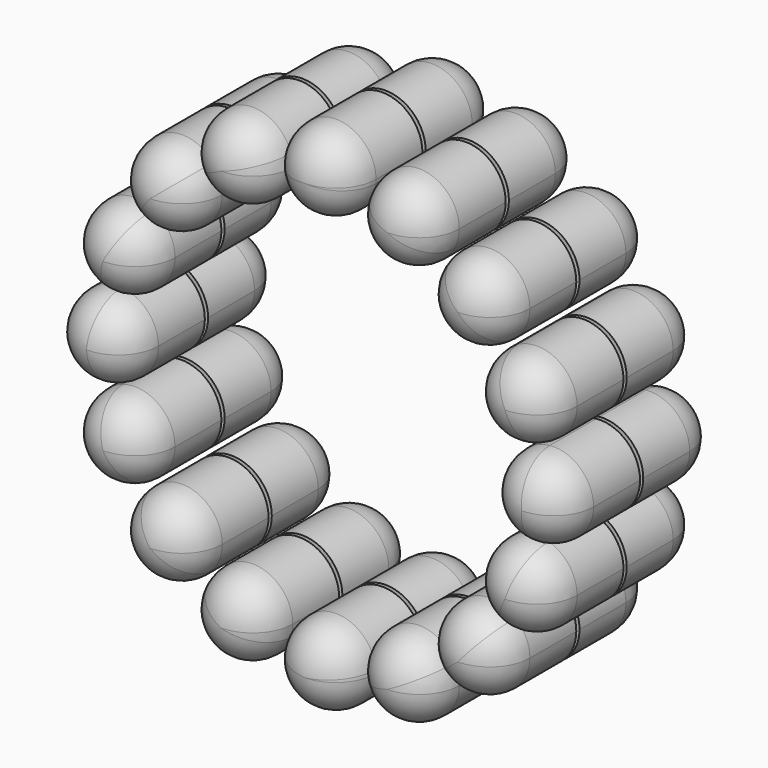
from build123d import *

# Parameters (mm, degrees)
F1_START      = 0.1
F1_DEPTH      = 4.9
F4_START      = -0.1
F4_DEPTH      = 4.9
F5_R          = 2
F5_2_R        = 2
F5_3_R        = 2
F5_4_R        = 2
F5_5_R        = 2
F5_6_R        = 2
F5_7_R        = 2
F5_8_R        = 2
F5_9_R        = 2
F5_10_R       = 2
F5_11_R       = 2
F5_12_R       = 2
F5_13_R       = 2
F5_14_R       = 2
F5_15_R       = 2
F5_16_R       = 2
F5_17_R       = 2
F5_18_R       = 2
F5_19_R       = 2
F5_20_R       = 2
F5_21_R       = 2
F5_22_R       = 2
F5_23_R       = 2
F5_24_R       = 2
F5_25_R       = 2
F5_26_R       = 2
F5_27_R       = 2
F5_28_R       = 2
F5_29_R       = 2
F5_30_R       = 2
F5_31_R       = 2
F5_32_R       = 2
F6_DEPTH      = 0.45
F6_DEPTH_BACK = 0.45


# Not quite as in the source:
# - the program builds the solid bodies; features that only make, move or delete a surface that nothing else refers to are left out


with BuildPart() as f1:
    # F0 (on Front) → F1 (new body)
    with BuildSketch(Plane.XZ.offset(F1_START)):
        with BuildLine():
            ThreePointArc((-1.9915265076, 10.691091954), (0, 8.875), (1.9915265076, 10.691091954))
            ThreePointArc((1.9915265076, 10.691091954), (1.793901159, 10.726021799), (1.5956648895, 10.7572988506))
            ThreePointArc((1.5956648895, 10.7572988506), (0, 9.275), (-1.5956648895, 10.7572988506))
            ThreePointArc((-1.5956648895, 10.7572988506), (-1.793901159, 10.726021799), (-1.9915265076, 10.691091954))
        make_face()
        with BuildLine():
            ThreePointArc((1.5956648895, 10.7572988506), (1.793901159, 10.726021799), (1.9915265076, 10.691091954))
            ThreePointArc((1.9915265076, 10.691091954), (1.9978805038, 10.7829484255), (2, 10.875))
            ThreePointArc((2, 10.875), (-0.0920515745, 12.8728805038), (-1.9915265076, 10.691091954))
            ThreePointArc((-1.9915265076, 10.691091954), (-1.793901159, 10.726021799), (-1.5956648895, 10.7572988506))
            ThreePointArc((-1.5956648895, 10.7572988506), (-0.0588904783, 12.4739158551), (1.6, 10.875))
            ThreePointArc((1.6, 10.875), (1.5989158551, 10.8161095217), (1.5956648895, 10.7572988506))
        make_face()
        with BuildLine():
            ThreePointArc((-1.5956648895, 10.7572988506), (0, 10.875), (1.5956648895, 10.7572988506))
            ThreePointArc((1.5956648895, 10.7572988506), (1.5989158551, 10.8161095217), (1.6, 10.875))
            ThreePointArc((1.6, 10.875), (-0.0588904783, 12.4739158551), (-1.5956648895, 10.7572988506))
        make_face()
        with BuildLine():
            ThreePointArc((-1.5956648895, 10.7572988506), (0, 9.275), (1.5956648895, 10.7572988506))
            ThreePointArc((1.5956648895, 10.7572988506), (0, 10.875), (-1.5956648895, 10.7572988506))
        make_face()
    extrude(amount=F1_DEPTH)

    # F5#3
    f5_3_edges = [f1.edges().sort_by_distance(p)[0] for p in [
        (-1.991527, -5, 11.058908),
    ]]
    fillet(f5_3_edges, radius=F5_3_R)


with BuildPart() as f1b:
    # F0 (on Front) → F1, piece 2 (new body)
    with BuildSketch(Plane.XZ.offset(F1_START)):
        with BuildLine():
            ThreePointArc((2.2513731858, 10.6394052361), (3.3963154622, 8.199430851), (5.9312343436, 9.1151568369))
            ThreePointArc((5.9312343436, 9.1151568369), (5.7620194018, 9.2230557525), (5.5908421792, 9.3278137164))
            ThreePointArc((5.5908421792, 9.3278137164), (3.5493888352, 8.568982664), (2.642437915, 10.54908275))
            ThreePointArc((2.642437915, 10.54908275), (2.4473222735, 10.5960482582), (2.2513731858, 10.6394052361))
        make_face()
        with BuildLine():
            ThreePointArc((5.5908421792, 9.3278137164), (5.7620194018, 9.2230557525), (5.9312343436, 9.1151568369))
            ThreePointArc((5.9312343436, 9.1151568369), (6.1032157458, 9.5671399359), (6.161682327, 10.0471899161))
            ThreePointArc((6.161682327, 10.0471899161), (4.4611666485, 12.0246400775), (2.2513731858, 10.6394052361))
            ThreePointArc((2.2513731858, 10.6394052361), (2.4473222735, 10.5960482582), (2.642437915, 10.54908275))
            ThreePointArc((2.642437915, 10.54908275), (4.4158564217, 11.6268720137), (5.761682327, 10.0471899161))
            ThreePointArc((5.761682327, 10.0471899161), (5.7183864998, 9.6774979927), (5.5908421792, 9.3278137164))
        make_face()
        with BuildLine():
            ThreePointArc((2.642437915, 10.54908275), (4.161682327, 10.0471899161), (5.5908421792, 9.3278137164))
            ThreePointArc((5.5908421792, 9.3278137164), (5.7183864998, 9.6774979927), (5.761682327, 10.0471899161))
            ThreePointArc((5.761682327, 10.0471899161), (4.4158564217, 11.6268720137), (2.642437915, 10.54908275))
        make_face()
        with BuildLine():
            ThreePointArc((2.642437915, 10.54908275), (3.5493888352, 8.568982664), (5.5908421792, 9.3278137164))
            ThreePointArc((5.5908421792, 9.3278137164), (4.161682327, 10.0471899161), (2.642437915, 10.54908275))
        make_face()
    extrude(amount=F1_DEPTH)

    # F5#4
    f5_4_edges = [f1b.edges().sort_by_distance(p)[0] for p in [
        (2.39213, -5, 10.979223),
    ]]
    fillet(f5_4_edges, radius=F5_4_R)


with BuildPart() as f1c:
    # F0 (on Front) → F1, piece 3 (new body)
    with BuildSketch(Plane.XZ.offset(F1_START)):
        with BuildLine():
            ThreePointArc((6.1515217205, 8.9679655174), (6.275572683, 6.275572683), (8.9679655174, 6.1515217205))
            ThreePointArc((8.9679655174, 6.1515217205), (8.8529224235, 6.3159630749), (8.7348644283, 6.4782535007))
            ThreePointArc((8.7348644283, 6.4782535007), (6.5584153955, 6.5584153955), (6.4782535007, 8.7348644283))
            ThreePointArc((6.4782535007, 8.7348644283), (6.3159630749, 8.8529224235), (6.1515217205, 8.9679655174))
        make_face()
        with BuildLine():
            ThreePointArc((8.7348644283, 6.4782535007), (8.8529224235, 6.3159630749), (8.9679655174, 6.1515217205))
            ThreePointArc((8.9679655174, 6.1515217205), (9.5003605388, 6.8401859112), (9.6897862454, 7.6897862454))
            ThreePointArc((9.6897862454, 7.6897862454), (8.3692974485, 9.5708137638), (6.1515217205, 8.9679655174))
            ThreePointArc((6.1515217205, 8.9679655174), (6.3159630749, 8.8529224235), (6.4782535007, 8.7348644283))
            ThreePointArc((6.4782535007, 8.7348644283), (8.2472571453, 9.1895282885), (9.2897862454, 7.6897862454))
            ThreePointArc((9.2897862454, 7.6897862454), (9.1444554677, 7.0234999303), (8.7348644283, 6.4782535007))
        make_face()
        with BuildLine():
            ThreePointArc((6.4782535007, 8.7348644283), (7.6897862454, 7.6897862454), (8.7348644283, 6.4782535007))
            ThreePointArc((8.7348644283, 6.4782535007), (9.1444554677, 7.0234999303), (9.2897862454, 7.6897862454))
            ThreePointArc((9.2897862454, 7.6897862454), (8.2472571453, 9.1895282885), (6.4782535007, 8.7348644283))
        make_face()
        with BuildLine():
            ThreePointArc((6.4782535007, 8.7348644283), (6.5584153955, 6.5584153955), (8.7348644283, 6.4782535007))
            ThreePointArc((8.7348644283, 6.4782535007), (7.6897862454, 7.6897862454), (6.4782535007, 8.7348644283))
        make_face()
    extrude(amount=F1_DEPTH)

    # F5#5
    f5_5_edges = [f1c.edges().sort_by_distance(p)[0] for p in [
        (6.411607, -5, 9.228051),
    ]]
    fillet(f5_5_edges, radius=F5_5_R)


with BuildPart() as f1d:
    # F0 (on Front) → F1, piece 4 (new body)
    with BuildSketch(Plane.XZ.offset(F1_START)):
        with BuildLine():
            ThreePointArc((9.1151568369, 5.9312343436), (8.199430851, 3.3963154622), (10.6394052361, 2.2513731858))
            ThreePointArc((10.6394052361, 2.2513731858), (10.5960482582, 2.4473222735), (10.54908275, 2.642437915))
            ThreePointArc((10.54908275, 2.642437915), (8.568982664, 3.5493888352), (9.3278137164, 5.5908421792))
            ThreePointArc((9.3278137164, 5.5908421792), (9.2230557525, 5.7620194018), (9.1151568369, 5.9312343436))
        make_face()
        with BuildLine():
            ThreePointArc((10.54908275, 2.642437915), (10.5960482582, 2.4473222735), (10.6394052361, 2.2513731858))
            ThreePointArc((10.6394052361, 2.2513731858), (11.6572257293, 2.975181303), (12.0471899161, 4.161682327))
            ThreePointArc((12.0471899161, 4.161682327), (11.0806147662, 5.8740003696), (9.1151568369, 5.9312343436))
            ThreePointArc((9.1151568369, 5.9312343436), (9.2230557525, 5.7620194018), (9.3278137164, 5.5908421792))
            ThreePointArc((9.3278137164, 5.5908421792), (10.886534327, 5.5238500699), (11.6471899161, 4.161682327))
            ThreePointArc((11.6471899161, 4.161682327), (11.3439220654, 3.2244066296), (10.54908275, 2.642437915))
        make_face()
        with BuildLine():
            ThreePointArc((9.3278137164, 5.5908421792), (10.0471899161, 4.161682327), (10.54908275, 2.642437915))
            ThreePointArc((10.54908275, 2.642437915), (11.3439220654, 3.2244066296), (11.6471899161, 4.161682327))
            ThreePointArc((11.6471899161, 4.161682327), (10.886534327, 5.5238500699), (9.3278137164, 5.5908421792))
        make_face()
        with BuildLine():
            ThreePointArc((9.3278137164, 5.5908421792), (8.568982664, 3.5493888352), (10.54908275, 2.642437915))
            ThreePointArc((10.54908275, 2.642437915), (10.0471899161, 4.161682327), (9.3278137164, 5.5908421792))
        make_face()
    extrude(amount=F1_DEPTH)

    # F5#6
    f5_6_edges = [f1d.edges().sort_by_distance(p)[0] for p in [
        (9.454975, -5, 6.071991),
    ]]
    fillet(f5_6_edges, radius=F5_6_R)


with BuildPart() as f1e:
    # F0 (on Front) → F1, piece 5 (new body)
    with BuildSketch(Plane.XZ.offset(F1_START)):
        with BuildLine():
            ThreePointArc((10.7572988506, -1.5956648895), (9.275, 0), (10.7572988506, 1.5956648895))
            ThreePointArc((10.7572988506, 1.5956648895), (10.726021799, 1.793901159), (10.691091954, 1.9915265076))
            ThreePointArc((10.691091954, 1.9915265076), (8.875, 0), (10.691091954, -1.9915265076))
            ThreePointArc((10.691091954, -1.9915265076), (10.726021799, -1.793901159), (10.7572988506, -1.5956648895))
        make_face()
        with BuildLine():
            ThreePointArc((10.691091954, 1.9915265076), (10.726021799, 1.793901159), (10.7572988506, 1.5956648895))
            ThreePointArc((10.7572988506, 1.5956648895), (11.9639623871, 1.1722461002), (12.475, 0))
            ThreePointArc((12.475, 0), (11.9639623871, -1.1722461002), (10.7572988506, -1.5956648895))
            ThreePointArc((10.7572988506, -1.5956648895), (10.726021799, -1.793901159), (10.691091954, -1.9915265076))
            ThreePointArc((10.691091954, -1.9915265076), (12.2226245597, -1.4778051448), (12.875, 0))
            ThreePointArc((12.875, 0), (12.2226245597, 1.4778051448), (10.691091954, 1.9915265076))
        make_face()
        with BuildLine():
            ThreePointArc((10.7572988506, 1.5956648895), (10.8455347955, 0.8), (10.875, 0))
            ThreePointArc((10.875, 0), (10.8455347955, -0.8), (10.7572988506, -1.5956648895))
            ThreePointArc((10.7572988506, -1.5956648895), (11.9639623871, -1.1722461002), (12.475, 0))
            ThreePointArc((12.475, 0), (11.9639623871, 1.1722461002), (10.7572988506, 1.5956648895))
        make_face()
        with BuildLine():
            ThreePointArc((10.7572988506, -1.5956648895), (10.8455347955, -0.8), (10.875, 0))
            ThreePointArc((10.875, 0), (10.8455347955, 0.8), (10.7572988506, 1.5956648895))
            ThreePointArc((10.7572988506, 1.5956648895), (9.275, 0), (10.7572988506, -1.5956648895))
        make_face()
    extrude(amount=F1_DEPTH)

    # F5#7
    f5_7_edges = [f1e.edges().sort_by_distance(p)[0] for p in [
        (11.058908, -5, 1.991527),
    ]]
    fillet(f5_7_edges, radius=F5_7_R)


with BuildPart() as f1f:
    # F0 (on Front) → F1, piece 6 (new body)
    with BuildSketch(Plane.XZ.offset(F1_START)):
        with BuildLine():
            ThreePointArc((10.54908275, -2.642437915), (10.5960482582, -2.4473222735), (10.6394052361, -2.2513731858))
            ThreePointArc((10.6394052361, -2.2513731858), (8.199430851, -3.3963154622), (9.1151568369, -5.9312343436))
            ThreePointArc((9.1151568369, -5.9312343436), (9.2230557525, -5.7620194018), (9.3278137164, -5.5908421792))
            ThreePointArc((9.3278137164, -5.5908421792), (8.568982664, -3.5493888352), (10.54908275, -2.642437915))
        make_face()
        with BuildLine():
            ThreePointArc((12.0471899161, -4.161682327), (11.6572257293, -2.975181303), (10.6394052361, -2.2513731858))
            ThreePointArc((10.6394052361, -2.2513731858), (10.5960482582, -2.4473222735), (10.54908275, -2.642437915))
            ThreePointArc((10.54908275, -2.642437915), (11.3439220654, -3.2244066296), (11.6471899161, -4.161682327))
            ThreePointArc((11.6471899161, -4.161682327), (10.886534327, -5.5238500699), (9.3278137164, -5.5908421792))
            ThreePointArc((9.3278137164, -5.5908421792), (9.2230557525, -5.7620194018), (9.1151568369, -5.9312343436))
            ThreePointArc((9.1151568369, -5.9312343436), (11.0806147662, -5.8740003696), (12.0471899161, -4.161682327))
        make_face()
        with BuildLine():
            ThreePointArc((11.6471899161, -4.161682327), (11.3439220654, -3.2244066296), (10.54908275, -2.642437915))
            ThreePointArc((10.54908275, -2.642437915), (10.0471899161, -4.161682327), (9.3278137164, -5.5908421792))
            ThreePointArc((9.3278137164, -5.5908421792), (10.886534327, -5.5238500699), (11.6471899161, -4.161682327))
        make_face()
        with BuildLine():
            ThreePointArc((9.3278137164, -5.5908421792), (10.0471899161, -4.161682327), (10.54908275, -2.642437915))
            ThreePointArc((10.54908275, -2.642437915), (8.568982664, -3.5493888352), (9.3278137164, -5.5908421792))
        make_face()
    extrude(amount=F1_DEPTH)

    # F5#8
    f5_8_edges = [f1f.edges().sort_by_distance(p)[0] for p in [
        (10.979223, -5, -2.39213),
    ]]
    fillet(f5_8_edges, radius=F5_8_R)


with BuildPart() as f1g:
    # F0 (on Front) → F1, piece 7 (new body)
    with BuildSketch(Plane.XZ.offset(F1_START)):
        with BuildLine():
            ThreePointArc((8.7348644283, -6.4782535007), (8.8529224235, -6.3159630749), (8.9679655174, -6.1515217205))
            ThreePointArc((8.9679655174, -6.1515217205), (6.275572683, -6.275572683), (6.1515217205, -8.9679655174))
            ThreePointArc((6.1515217205, -8.9679655174), (6.3159630749, -8.8529224235), (6.4782535007, -8.7348644283))
            ThreePointArc((6.4782535007, -8.7348644283), (6.5584153955, -6.5584153955), (8.7348644283, -6.4782535007))
        make_face()
        with BuildLine():
            ThreePointArc((9.6897862454, -7.6897862454), (9.5003605388, -6.8401859112), (8.9679655174, -6.1515217205))
            ThreePointArc((8.9679655174, -6.1515217205), (8.8529224235, -6.3159630749), (8.7348644283, -6.4782535007))
            ThreePointArc((8.7348644283, -6.4782535007), (9.1444554677, -7.0234999303), (9.2897862454, -7.6897862454))
            ThreePointArc((9.2897862454, -7.6897862454), (8.2472571453, -9.1895282885), (6.4782535007, -8.7348644283))
            ThreePointArc((6.4782535007, -8.7348644283), (6.3159630749, -8.8529224235), (6.1515217205, -8.9679655174))
            ThreePointArc((6.1515217205, -8.9679655174), (8.3692974485, -9.5708137638), (9.6897862454, -7.6897862454))
        make_face()
        with BuildLine():
            ThreePointArc((9.2897862454, -7.6897862454), (9.1444554677, -7.0234999303), (8.7348644283, -6.4782535007))
            ThreePointArc((8.7348644283, -6.4782535007), (7.6897862454, -7.6897862454), (6.4782535007, -8.7348644283))
            ThreePointArc((6.4782535007, -8.7348644283), (8.2472571453, -9.1895282885), (9.2897862454, -7.6897862454))
        make_face()
        with BuildLine():
            ThreePointArc((6.4782535007, -8.7348644283), (7.6897862454, -7.6897862454), (8.7348644283, -6.4782535007))
            ThreePointArc((8.7348644283, -6.4782535007), (6.5584153955, -6.5584153955), (6.4782535007, -8.7348644283))
        make_face()
    extrude(amount=F1_DEPTH)

    # F5#9
    f5_9_edges = [f1g.edges().sort_by_distance(p)[0] for p in [
        (9.228051, -5, -6.411607),
    ]]
    fillet(f5_9_edges, radius=F5_9_R)


with BuildPart() as f1h:
    # F0 (on Front) → F1, piece 8 (new body)
    with BuildSketch(Plane.XZ.offset(F1_START)):
        with BuildLine():
            ThreePointArc((5.5908421792, -9.3278137164), (5.7620194018, -9.2230557525), (5.9312343436, -9.1151568369))
            ThreePointArc((5.9312343436, -9.1151568369), (3.3963154622, -8.199430851), (2.2513731858, -10.6394052361))
            ThreePointArc((2.2513731858, -10.6394052361), (2.4473222735, -10.5960482582), (2.642437915, -10.54908275))
            ThreePointArc((2.642437915, -10.54908275), (3.5493888352, -8.568982664), (5.5908421792, -9.3278137164))
        make_face()
        with BuildLine():
            ThreePointArc((6.161682327, -10.0471899161), (6.1032157458, -9.5671399359), (5.9312343436, -9.1151568369))
            ThreePointArc((5.9312343436, -9.1151568369), (5.7620194018, -9.2230557525), (5.5908421792, -9.3278137164))
            ThreePointArc((5.5908421792, -9.3278137164), (5.7183864998, -9.6774979927), (5.761682327, -10.0471899161))
            ThreePointArc((5.761682327, -10.0471899161), (4.4158564217, -11.6268720137), (2.642437915, -10.54908275))
            ThreePointArc((2.642437915, -10.54908275), (2.4473222735, -10.5960482582), (2.2513731858, -10.6394052361))
            ThreePointArc((2.2513731858, -10.6394052361), (4.4611666485, -12.0246400775), (6.161682327, -10.0471899161))
        make_face()
        with BuildLine():
            ThreePointArc((5.761682327, -10.0471899161), (5.7183864998, -9.6774979927), (5.5908421792, -9.3278137164))
            ThreePointArc((5.5908421792, -9.3278137164), (4.161682327, -10.0471899161), (2.642437915, -10.54908275))
            ThreePointArc((2.642437915, -10.54908275), (4.4158564217, -11.6268720137), (5.761682327, -10.0471899161))
        make_face()
        with BuildLine():
            ThreePointArc((2.642437915, -10.54908275), (4.161682327, -10.0471899161), (5.5908421792, -9.3278137164))
            ThreePointArc((5.5908421792, -9.3278137164), (3.5493888352, -8.568982664), (2.642437915, -10.54908275))
        make_face()
    extrude(amount=F1_DEPTH)

    # F5#10
    f5_10_edges = [f1h.edges().sort_by_distance(p)[0] for p in [
        (6.071991, -5, -9.454975),
    ]]
    fillet(f5_10_edges, radius=F5_10_R)


with BuildPart() as f1i:
    # F0 (on Front) → F1, piece 9 (new body)
    with BuildSketch(Plane.XZ.offset(F1_START)):
        with BuildLine():
            ThreePointArc((1.5956648895, -10.7572988506), (1.793901159, -10.726021799), (1.9915265076, -10.691091954))
            ThreePointArc((1.9915265076, -10.691091954), (0, -8.875), (-1.9915265076, -10.691091954))
            ThreePointArc((-1.9915265076, -10.691091954), (-1.793901159, -10.726021799), (-1.5956648895, -10.7572988506))
            ThreePointArc((-1.5956648895, -10.7572988506), (0, -9.275), (1.5956648895, -10.7572988506))
        make_face()
        with BuildLine():
            ThreePointArc((2, -10.875), (1.9978805038, -10.7829484255), (1.9915265076, -10.691091954))
            ThreePointArc((1.9915265076, -10.691091954), (1.793901159, -10.726021799), (1.5956648895, -10.7572988506))
            ThreePointArc((1.5956648895, -10.7572988506), (1.5989158551, -10.8161095217), (1.6, -10.875))
            ThreePointArc((1.6, -10.875), (-0.0588904783, -12.4739158551), (-1.5956648895, -10.7572988506))
            ThreePointArc((-1.5956648895, -10.7572988506), (-1.793901159, -10.726021799), (-1.9915265076, -10.691091954))
            ThreePointArc((-1.9915265076, -10.691091954), (-0.0920515745, -12.8728805038), (2, -10.875))
        make_face()
        with BuildLine():
            ThreePointArc((1.6, -10.875), (1.5989158551, -10.8161095217), (1.5956648895, -10.7572988506))
            ThreePointArc((1.5956648895, -10.7572988506), (0, -10.875), (-1.5956648895, -10.7572988506))
            ThreePointArc((-1.5956648895, -10.7572988506), (-0.0588904783, -12.4739158551), (1.6, -10.875))
        make_face()
        with BuildLine():
            ThreePointArc((-1.5956648895, -10.7572988506), (0, -10.875), (1.5956648895, -10.7572988506))
            ThreePointArc((1.5956648895, -10.7572988506), (0, -9.275), (-1.5956648895, -10.7572988506))
        make_face()
    extrude(amount=F1_DEPTH)

    # F5#11
    f5_11_edges = [f1i.edges().sort_by_distance(p)[0] for p in [
        (1.991527, -5, -11.058908),
    ]]
    fillet(f5_11_edges, radius=F5_11_R)


with BuildPart() as f1j:
    # F0 (on Front) → F1, piece 10 (new body)
    with BuildSketch(Plane.XZ.offset(F1_START)):
        with BuildLine():
            ThreePointArc((-5.9312343436, -9.1151568369), (-4.9270491917, -11.8949489811), (-2.2513731858, -10.6394052361))
            ThreePointArc((-2.2513731858, -10.6394052361), (-2.4473222735, -10.5960482582), (-2.642437915, -10.54908275))
            ThreePointArc((-2.642437915, -10.54908275), (-4.7739758188, -11.5253971681), (-5.5908421792, -9.3278137164))
            ThreePointArc((-5.5908421792, -9.3278137164), (-5.7620194018, -9.2230557525), (-5.9312343436, -9.1151568369))
        make_face()
        with BuildLine():
            ThreePointArc((-2.642437915, -10.54908275), (-2.4473222735, -10.5960482582), (-2.2513731858, -10.6394052361))
            ThreePointArc((-2.2513731858, -10.6394052361), (-2.1842321655, -10.3466742376), (-2.161682327, -10.0471899161))
            ThreePointArc((-2.161682327, -10.0471899161), (-3.6816323468, -8.1056564972), (-5.9312343436, -9.1151568369))
            ThreePointArc((-5.9312343436, -9.1151568369), (-5.7620194018, -9.2230557525), (-5.5908421792, -9.3278137164))
            ThreePointArc((-5.5908421792, -9.3278137164), (-3.7919904036, -8.4904857432), (-2.561682327, -10.0471899161))
            ThreePointArc((-2.561682327, -10.0471899161), (-2.5820002293, -10.3013640108), (-2.642437915, -10.54908275))
        make_face()
        with BuildLine():
            ThreePointArc((-5.5908421792, -9.3278137164), (-4.7739758188, -11.5253971681), (-2.642437915, -10.54908275))
            ThreePointArc((-2.642437915, -10.54908275), (-4.161682327, -10.0471899161), (-5.5908421792, -9.3278137164))
        make_face()
        with BuildLine():
            ThreePointArc((-5.5908421792, -9.3278137164), (-4.161682327, -10.0471899161), (-2.642437915, -10.54908275))
            ThreePointArc((-2.642437915, -10.54908275), (-2.5820002293, -10.3013640108), (-2.561682327, -10.0471899161))
            ThreePointArc((-2.561682327, -10.0471899161), (-3.7919904036, -8.4904857432), (-5.5908421792, -9.3278137164))
        make_face()
    extrude(amount=F1_DEPTH)

    # F5#12
    f5_12_edges = [f1j.edges().sort_by_distance(p)[0] for p in [
        (-6.071991, -5, -9.454975),
    ]]
    fillet(f5_12_edges, radius=F5_12_R)


with BuildPart() as f1k:
    # F0 (on Front) → F1, piece 11 (new body)
    with BuildSketch(Plane.XZ.offset(F1_START)):
        with BuildLine():
            ThreePointArc((-8.9679655174, -6.1515217205), (-9.1039998078, -9.1039998078), (-6.1515217205, -8.9679655174))
            ThreePointArc((-6.1515217205, -8.9679655174), (-6.3159630749, -8.8529224235), (-6.4782535007, -8.7348644283))
            ThreePointArc((-6.4782535007, -8.7348644283), (-8.8211570953, -8.8211570953), (-8.7348644283, -6.4782535007))
            ThreePointArc((-8.7348644283, -6.4782535007), (-8.8529224235, -6.3159630749), (-8.9679655174, -6.1515217205))
        make_face()
        with BuildLine():
            ThreePointArc((-6.4782535007, -8.7348644283), (-6.3159630749, -8.8529224235), (-6.1515217205, -8.9679655174))
            ThreePointArc((-6.1515217205, -8.9679655174), (-5.808758727, -8.3692974485), (-5.6897862454, -7.6897862454))
            ThreePointArc((-5.6897862454, -7.6897862454), (-6.8401859112, -5.879211952), (-8.9679655174, -6.1515217205))
            ThreePointArc((-8.9679655174, -6.1515217205), (-8.8529224235, -6.3159630749), (-8.7348644283, -6.4782535007))
            ThreePointArc((-8.7348644283, -6.4782535007), (-7.0234999303, -6.2351170231), (-6.0897862454, -7.6897862454))
            ThreePointArc((-6.0897862454, -7.6897862454), (-6.1900442023, -8.2472571453), (-6.4782535007, -8.7348644283))
        make_face()
        with BuildLine():
            ThreePointArc((-8.7348644283, -6.4782535007), (-8.8211570953, -8.8211570953), (-6.4782535007, -8.7348644283))
            ThreePointArc((-6.4782535007, -8.7348644283), (-7.6897862454, -7.6897862454), (-8.7348644283, -6.4782535007))
        make_face()
        with BuildLine():
            ThreePointArc((-8.7348644283, -6.4782535007), (-7.6897862454, -7.6897862454), (-6.4782535007, -8.7348644283))
            ThreePointArc((-6.4782535007, -8.7348644283), (-6.1900442023, -8.2472571453), (-6.0897862454, -7.6897862454))
            ThreePointArc((-6.0897862454, -7.6897862454), (-7.0234999303, -6.2351170231), (-8.7348644283, -6.4782535007))
        make_face()
    extrude(amount=F1_DEPTH)

    # F5#13
    f5_13_edges = [f1k.edges().sort_by_distance(p)[0] for p in [
        (-9.228051, -5, -6.411607),
    ]]
    fillet(f5_13_edges, radius=F5_13_R)


with BuildPart() as f1l:
    # F0 (on Front) → F1, piece 12 (new body)
    with BuildSketch(Plane.XZ.offset(F1_START)):
        with BuildLine():
            ThreePointArc((-10.6394052361, -2.2513731858), (-11.8949489811, -4.9270491917), (-9.1151568369, -5.9312343436))
            ThreePointArc((-9.1151568369, -5.9312343436), (-9.2230557525, -5.7620194018), (-9.3278137164, -5.5908421792))
            ThreePointArc((-9.3278137164, -5.5908421792), (-11.5253971681, -4.7739758188), (-10.54908275, -2.642437915))
            ThreePointArc((-10.54908275, -2.642437915), (-10.5960482582, -2.4473222735), (-10.6394052361, -2.2513731858))
        make_face()
        with BuildLine():
            ThreePointArc((-9.3278137164, -5.5908421792), (-9.2230557525, -5.7620194018), (-9.1151568369, -5.9312343436))
            ThreePointArc((-9.1151568369, -5.9312343436), (-8.3348718734, -5.1951071771), (-8.0471899161, -4.161682327))
            ThreePointArc((-8.0471899161, -4.161682327), (-8.8606888921, -2.5516465137), (-10.6394052361, -2.2513731858))
            ThreePointArc((-10.6394052361, -2.2513731858), (-10.5960482582, -2.4473222735), (-10.54908275, -2.642437915))
            ThreePointArc((-10.54908275, -2.642437915), (-9.1099142187, -2.8649501776), (-8.4471899161, -4.161682327))
            ThreePointArc((-8.4471899161, -4.161682327), (-8.6850221732, -5.0010267379), (-9.3278137164, -5.5908421792))
        make_face()
        with BuildLine():
            ThreePointArc((-10.54908275, -2.642437915), (-11.5253971681, -4.7739758188), (-9.3278137164, -5.5908421792))
            ThreePointArc((-9.3278137164, -5.5908421792), (-10.0471899161, -4.161682327), (-10.54908275, -2.642437915))
        make_face()
        with BuildLine():
            ThreePointArc((-10.54908275, -2.642437915), (-10.0471899161, -4.161682327), (-9.3278137164, -5.5908421792))
            ThreePointArc((-9.3278137164, -5.5908421792), (-8.6850221732, -5.0010267379), (-8.4471899161, -4.161682327))
            ThreePointArc((-8.4471899161, -4.161682327), (-9.1099142187, -2.8649501776), (-10.54908275, -2.642437915))
        make_face()
    extrude(amount=F1_DEPTH)

    # F5#14
    f5_14_edges = [f1l.edges().sort_by_distance(p)[0] for p in [
        (-10.979223, -5, -2.39213),
    ]]
    fillet(f5_14_edges, radius=F5_14_R)


with BuildPart() as f1m:
    # F0 (on Front) → F1, piece 13 (new body)
    with BuildSketch(Plane.XZ.offset(F1_START)):
        with BuildLine():
            ThreePointArc((-10.7572988506, 1.5956648895), (-10.726021799, 1.793901159), (-10.691091954, 1.9915265076))
            ThreePointArc((-10.691091954, 1.9915265076), (-12.875, 0), (-10.691091954, -1.9915265076))
            ThreePointArc((-10.691091954, -1.9915265076), (-10.726021799, -1.793901159), (-10.7572988506, -1.5956648895))
            ThreePointArc((-10.7572988506, -1.5956648895), (-12.475, 0), (-10.7572988506, 1.5956648895))
        make_face()
        with BuildLine():
            ThreePointArc((-8.875, 0), (-9.3971948552, 1.3476245597), (-10.691091954, 1.9915265076))
            ThreePointArc((-10.691091954, 1.9915265076), (-10.726021799, 1.793901159), (-10.7572988506, 1.5956648895))
            ThreePointArc((-10.7572988506, 1.5956648895), (-9.7027538998, 1.0889623871), (-9.275, 0))
            ThreePointArc((-9.275, 0), (-9.7027538998, -1.0889623871), (-10.7572988506, -1.5956648895))
            ThreePointArc((-10.7572988506, -1.5956648895), (-10.726021799, -1.793901159), (-10.691091954, -1.9915265076))
            ThreePointArc((-10.691091954, -1.9915265076), (-9.3971948552, -1.3476245597), (-8.875, 0))
        make_face()
        with BuildLine():
            ThreePointArc((-10.7572988506, -1.5956648895), (-10.875, 0), (-10.7572988506, 1.5956648895))
            ThreePointArc((-10.7572988506, 1.5956648895), (-12.475, 0), (-10.7572988506, -1.5956648895))
        make_face()
        with BuildLine():
            ThreePointArc((-9.275, 0), (-9.7027538998, 1.0889623871), (-10.7572988506, 1.5956648895))
            ThreePointArc((-10.7572988506, 1.5956648895), (-10.875, 0), (-10.7572988506, -1.5956648895))
            ThreePointArc((-10.7572988506, -1.5956648895), (-9.7027538998, -1.0889623871), (-9.275, 0))
        make_face()
    extrude(amount=F1_DEPTH)

    # F5#15
    f5_15_edges = [f1m.edges().sort_by_distance(p)[0] for p in [
        (-11.058908, -5, 1.991527),
    ]]
    fillet(f5_15_edges, radius=F5_15_R)


with BuildPart() as f1n:
    # F0 (on Front) → F1, piece 14 (new body)
    with BuildSketch(Plane.XZ.offset(F1_START)):
        with BuildLine():
            ThreePointArc((-9.3278137164, 5.5908421792), (-9.2230557525, 5.7620194018), (-9.1151568369, 5.9312343436))
            ThreePointArc((-9.1151568369, 5.9312343436), (-11.8949489811, 4.9270491917), (-10.6394052361, 2.2513731858))
            ThreePointArc((-10.6394052361, 2.2513731858), (-10.5960482582, 2.4473222735), (-10.54908275, 2.642437915))
            ThreePointArc((-10.54908275, 2.642437915), (-11.5253971681, 4.7739758188), (-9.3278137164, 5.5908421792))
        make_face()
        with BuildLine():
            ThreePointArc((-8.0471899161, 4.161682327), (-8.3348718734, 5.1951071771), (-9.1151568369, 5.9312343436))
            ThreePointArc((-9.1151568369, 5.9312343436), (-9.2230557525, 5.7620194018), (-9.3278137164, 5.5908421792))
            ThreePointArc((-9.3278137164, 5.5908421792), (-8.6850221732, 5.0010267379), (-8.4471899161, 4.161682327))
            ThreePointArc((-8.4471899161, 4.161682327), (-9.1099142187, 2.8649501776), (-10.54908275, 2.642437915))
            ThreePointArc((-10.54908275, 2.642437915), (-10.5960482582, 2.4473222735), (-10.6394052361, 2.2513731858))
            ThreePointArc((-10.6394052361, 2.2513731858), (-8.8606888921, 2.5516465137), (-8.0471899161, 4.161682327))
        make_face()
        with BuildLine():
            ThreePointArc((-10.54908275, 2.642437915), (-10.0471899161, 4.161682327), (-9.3278137164, 5.5908421792))
            ThreePointArc((-9.3278137164, 5.5908421792), (-11.5253971681, 4.7739758188), (-10.54908275, 2.642437915))
        make_face()
        with BuildLine():
            ThreePointArc((-8.4471899161, 4.161682327), (-8.6850221732, 5.0010267379), (-9.3278137164, 5.5908421792))
            ThreePointArc((-9.3278137164, 5.5908421792), (-10.0471899161, 4.161682327), (-10.54908275, 2.642437915))
            ThreePointArc((-10.54908275, 2.642437915), (-9.1099142187, 2.8649501776), (-8.4471899161, 4.161682327))
        make_face()
    extrude(amount=F1_DEPTH)

    # F5#16
    f5_16_edges = [f1n.edges().sort_by_distance(p)[0] for p in [
        (-9.454975, -5, 6.071991),
    ]]
    fillet(f5_16_edges, radius=F5_16_R)


with BuildPart() as f1o:
    # F0 (on Front) → F1, piece 15 (new body)
    with BuildSketch(Plane.XZ.offset(F1_START)):
        with BuildLine():
            ThreePointArc((-6.4782535007, 8.7348644283), (-6.3159630749, 8.8529224235), (-6.1515217205, 8.9679655174))
            ThreePointArc((-6.1515217205, 8.9679655174), (-9.1039998078, 9.1039998078), (-8.9679655174, 6.1515217205))
            ThreePointArc((-8.9679655174, 6.1515217205), (-8.8529224235, 6.3159630749), (-8.7348644283, 6.4782535007))
            ThreePointArc((-8.7348644283, 6.4782535007), (-8.8211570953, 8.8211570953), (-6.4782535007, 8.7348644283))
        make_face()
        with BuildLine():
            ThreePointArc((-5.6897862454, 7.6897862454), (-5.808758727, 8.3692974485), (-6.1515217205, 8.9679655174))
            ThreePointArc((-6.1515217205, 8.9679655174), (-6.3159630749, 8.8529224235), (-6.4782535007, 8.7348644283))
            ThreePointArc((-6.4782535007, 8.7348644283), (-6.1900442023, 8.2472571453), (-6.0897862454, 7.6897862454))
            ThreePointArc((-6.0897862454, 7.6897862454), (-7.0234999303, 6.2351170231), (-8.7348644283, 6.4782535007))
            ThreePointArc((-8.7348644283, 6.4782535007), (-8.8529224235, 6.3159630749), (-8.9679655174, 6.1515217205))
            ThreePointArc((-8.9679655174, 6.1515217205), (-6.8401859112, 5.879211952), (-5.6897862454, 7.6897862454))
        make_face()
        with BuildLine():
            ThreePointArc((-8.7348644283, 6.4782535007), (-7.6897862454, 7.6897862454), (-6.4782535007, 8.7348644283))
            ThreePointArc((-6.4782535007, 8.7348644283), (-8.8211570953, 8.8211570953), (-8.7348644283, 6.4782535007))
        make_face()
        with BuildLine():
            ThreePointArc((-6.0897862454, 7.6897862454), (-6.1900442023, 8.2472571453), (-6.4782535007, 8.7348644283))
            ThreePointArc((-6.4782535007, 8.7348644283), (-7.6897862454, 7.6897862454), (-8.7348644283, 6.4782535007))
            ThreePointArc((-8.7348644283, 6.4782535007), (-7.0234999303, 6.2351170231), (-6.0897862454, 7.6897862454))
        make_face()
    extrude(amount=F1_DEPTH)

    # F5
    f5_edges = [f1o.edges().sort_by_distance(p)[0] for p in [
        (-6.411607, -5, 9.228051),
    ]]
    fillet(f5_edges, radius=F5_R)


with BuildPart() as f1p:
    # F0 (on Front) → F1, piece 16 (new body)
    with BuildSketch(Plane.XZ.offset(F1_START)):
        with BuildLine():
            ThreePointArc((-2.642437915, 10.54908275), (-2.4473222735, 10.5960482582), (-2.2513731858, 10.6394052361))
            ThreePointArc((-2.2513731858, 10.6394052361), (-4.9270491917, 11.8949489811), (-5.9312343436, 9.1151568369))
            ThreePointArc((-5.9312343436, 9.1151568369), (-5.7620194018, 9.2230557525), (-5.5908421792, 9.3278137164))
            ThreePointArc((-5.5908421792, 9.3278137164), (-4.7739758188, 11.5253971681), (-2.642437915, 10.54908275))
        make_face()
        with BuildLine():
            ThreePointArc((-2.161682327, 10.0471899161), (-2.1842321655, 10.3466742376), (-2.2513731858, 10.6394052361))
            ThreePointArc((-2.2513731858, 10.6394052361), (-2.4473222735, 10.5960482582), (-2.642437915, 10.54908275))
            ThreePointArc((-2.642437915, 10.54908275), (-2.5820002293, 10.3013640108), (-2.561682327, 10.0471899161))
            ThreePointArc((-2.561682327, 10.0471899161), (-3.7919904036, 8.4904857432), (-5.5908421792, 9.3278137164))
            ThreePointArc((-5.5908421792, 9.3278137164), (-5.7620194018, 9.2230557525), (-5.9312343436, 9.1151568369))
            ThreePointArc((-5.9312343436, 9.1151568369), (-3.6816323468, 8.1056564972), (-2.161682327, 10.0471899161))
        make_face()
        with BuildLine():
            ThreePointArc((-5.5908421792, 9.3278137164), (-4.161682327, 10.0471899161), (-2.642437915, 10.54908275))
            ThreePointArc((-2.642437915, 10.54908275), (-4.7739758188, 11.5253971681), (-5.5908421792, 9.3278137164))
        make_face()
        with BuildLine():
            ThreePointArc((-2.561682327, 10.0471899161), (-2.5820002293, 10.3013640108), (-2.642437915, 10.54908275))
            ThreePointArc((-2.642437915, 10.54908275), (-4.161682327, 10.0471899161), (-5.5908421792, 9.3278137164))
            ThreePointArc((-5.5908421792, 9.3278137164), (-3.7919904036, 8.4904857432), (-2.561682327, 10.0471899161))
        make_face()
    extrude(amount=F1_DEPTH)

    # F5#2
    f5_2_edges = [f1p.edges().sort_by_distance(p)[0] for p in [
        (-2.39213, -5, 10.979223),
    ]]
    fillet(f5_2_edges, radius=F5_2_R)


with BuildPart() as f4:
    # F0 (on Front) → F4 (new body)
    with BuildSketch(Plane.XZ.offset(F4_START)):
        with BuildLine():
            ThreePointArc((11.6471899161, -4.161682327), (11.3439220654, -3.2244066296), (10.54908275, -2.642437915))
            ThreePointArc((10.54908275, -2.642437915), (10.0471899161, -4.161682327), (9.3278137164, -5.5908421792))
            ThreePointArc((9.3278137164, -5.5908421792), (10.886534327, -5.5238500699), (11.6471899161, -4.161682327))
        make_face()
        with BuildLine():
            ThreePointArc((12.0471899161, -4.161682327), (11.6572257293, -2.975181303), (10.6394052361, -2.2513731858))
            ThreePointArc((10.6394052361, -2.2513731858), (10.5960482582, -2.4473222735), (10.54908275, -2.642437915))
            ThreePointArc((10.54908275, -2.642437915), (11.3439220654, -3.2244066296), (11.6471899161, -4.161682327))
            ThreePointArc((11.6471899161, -4.161682327), (10.886534327, -5.5238500699), (9.3278137164, -5.5908421792))
            ThreePointArc((9.3278137164, -5.5908421792), (9.2230557525, -5.7620194018), (9.1151568369, -5.9312343436))
            ThreePointArc((9.1151568369, -5.9312343436), (11.0806147662, -5.8740003696), (12.0471899161, -4.161682327))
        make_face()
        with BuildLine():
            ThreePointArc((9.3278137164, -5.5908421792), (10.0471899161, -4.161682327), (10.54908275, -2.642437915))
            ThreePointArc((10.54908275, -2.642437915), (8.568982664, -3.5493888352), (9.3278137164, -5.5908421792))
        make_face()
        with BuildLine():
            ThreePointArc((10.54908275, -2.642437915), (10.5960482582, -2.4473222735), (10.6394052361, -2.2513731858))
            ThreePointArc((10.6394052361, -2.2513731858), (8.199430851, -3.3963154622), (9.1151568369, -5.9312343436))
            ThreePointArc((9.1151568369, -5.9312343436), (9.2230557525, -5.7620194018), (9.3278137164, -5.5908421792))
            ThreePointArc((9.3278137164, -5.5908421792), (8.568982664, -3.5493888352), (10.54908275, -2.642437915))
        make_face()
    extrude(amount=-F4_DEPTH)

    # F5#29
    f5_29_edges = [f4.edges().sort_by_distance(p)[0] for p in [
        (9.454975, 5, -6.071991),
    ]]
    fillet(f5_29_edges, radius=F5_29_R)


with BuildPart() as f4b:
    # F0 (on Front) → F4, piece 2 (new body)
    with BuildSketch(Plane.XZ.offset(F4_START)):
        with BuildLine():
            ThreePointArc((8.7348644283, -6.4782535007), (8.8529224235, -6.3159630749), (8.9679655174, -6.1515217205))
            ThreePointArc((8.9679655174, -6.1515217205), (6.275572683, -6.275572683), (6.1515217205, -8.9679655174))
            ThreePointArc((6.1515217205, -8.9679655174), (6.3159630749, -8.8529224235), (6.4782535007, -8.7348644283))
            ThreePointArc((6.4782535007, -8.7348644283), (6.5584153955, -6.5584153955), (8.7348644283, -6.4782535007))
        make_face()
        with BuildLine():
            ThreePointArc((6.4782535007, -8.7348644283), (7.6897862454, -7.6897862454), (8.7348644283, -6.4782535007))
            ThreePointArc((8.7348644283, -6.4782535007), (6.5584153955, -6.5584153955), (6.4782535007, -8.7348644283))
        make_face()
        with BuildLine():
            ThreePointArc((9.2897862454, -7.6897862454), (9.1444554677, -7.0234999303), (8.7348644283, -6.4782535007))
            ThreePointArc((8.7348644283, -6.4782535007), (7.6897862454, -7.6897862454), (6.4782535007, -8.7348644283))
            ThreePointArc((6.4782535007, -8.7348644283), (8.2472571453, -9.1895282885), (9.2897862454, -7.6897862454))
        make_face()
        with BuildLine():
            ThreePointArc((9.6897862454, -7.6897862454), (9.5003605388, -6.8401859112), (8.9679655174, -6.1515217205))
            ThreePointArc((8.9679655174, -6.1515217205), (8.8529224235, -6.3159630749), (8.7348644283, -6.4782535007))
            ThreePointArc((8.7348644283, -6.4782535007), (9.1444554677, -7.0234999303), (9.2897862454, -7.6897862454))
            ThreePointArc((9.2897862454, -7.6897862454), (8.2472571453, -9.1895282885), (6.4782535007, -8.7348644283))
            ThreePointArc((6.4782535007, -8.7348644283), (6.3159630749, -8.8529224235), (6.1515217205, -8.9679655174))
            ThreePointArc((6.1515217205, -8.9679655174), (8.3692974485, -9.5708137638), (9.6897862454, -7.6897862454))
        make_face()
    extrude(amount=-F4_DEPTH)

    # F5#28
    f5_28_edges = [f4b.edges().sort_by_distance(p)[0] for p in [
        (9.228051, 5, -6.411607),
    ]]
    fillet(f5_28_edges, radius=F5_28_R)


with BuildPart() as f4c:
    # F0 (on Front) → F4, piece 3 (new body)
    with BuildSketch(Plane.XZ.offset(F4_START)):
        with BuildLine():
            ThreePointArc((6.161682327, -10.0471899161), (6.1032157458, -9.5671399359), (5.9312343436, -9.1151568369))
            ThreePointArc((5.9312343436, -9.1151568369), (5.7620194018, -9.2230557525), (5.5908421792, -9.3278137164))
            ThreePointArc((5.5908421792, -9.3278137164), (5.7183864998, -9.6774979927), (5.761682327, -10.0471899161))
            ThreePointArc((5.761682327, -10.0471899161), (4.4158564217, -11.6268720137), (2.642437915, -10.54908275))
            ThreePointArc((2.642437915, -10.54908275), (2.4473222735, -10.5960482582), (2.2513731858, -10.6394052361))
            ThreePointArc((2.2513731858, -10.6394052361), (4.4611666485, -12.0246400775), (6.161682327, -10.0471899161))
        make_face()
        with BuildLine():
            ThreePointArc((5.761682327, -10.0471899161), (5.7183864998, -9.6774979927), (5.5908421792, -9.3278137164))
            ThreePointArc((5.5908421792, -9.3278137164), (4.161682327, -10.0471899161), (2.642437915, -10.54908275))
            ThreePointArc((2.642437915, -10.54908275), (4.4158564217, -11.6268720137), (5.761682327, -10.0471899161))
        make_face()
        with BuildLine():
            ThreePointArc((2.642437915, -10.54908275), (4.161682327, -10.0471899161), (5.5908421792, -9.3278137164))
            ThreePointArc((5.5908421792, -9.3278137164), (3.5493888352, -8.568982664), (2.642437915, -10.54908275))
        make_face()
        with BuildLine():
            ThreePointArc((5.5908421792, -9.3278137164), (5.7620194018, -9.2230557525), (5.9312343436, -9.1151568369))
            ThreePointArc((5.9312343436, -9.1151568369), (3.3963154622, -8.199430851), (2.2513731858, -10.6394052361))
            ThreePointArc((2.2513731858, -10.6394052361), (2.4473222735, -10.5960482582), (2.642437915, -10.54908275))
            ThreePointArc((2.642437915, -10.54908275), (3.5493888352, -8.568982664), (5.5908421792, -9.3278137164))
        make_face()
    extrude(amount=-F4_DEPTH)

    # F5#27
    f5_27_edges = [f4c.edges().sort_by_distance(p)[0] for p in [
        (2.39213, 5, -10.979223),
    ]]
    fillet(f5_27_edges, radius=F5_27_R)


with BuildPart() as f4d:
    # F0 (on Front) → F4, piece 4 (new body)
    with BuildSketch(Plane.XZ.offset(F4_START)):
        with BuildLine():
            ThreePointArc((-1.5956648895, -10.7572988506), (0, -10.875), (1.5956648895, -10.7572988506))
            ThreePointArc((1.5956648895, -10.7572988506), (0, -9.275), (-1.5956648895, -10.7572988506))
        make_face()
        with BuildLine():
            ThreePointArc((1.6, -10.875), (1.5989158551, -10.8161095217), (1.5956648895, -10.7572988506))
            ThreePointArc((1.5956648895, -10.7572988506), (0, -10.875), (-1.5956648895, -10.7572988506))
            ThreePointArc((-1.5956648895, -10.7572988506), (-0.0588904783, -12.4739158551), (1.6, -10.875))
        make_face()
        with BuildLine():
            ThreePointArc((2, -10.875), (1.9978805038, -10.7829484255), (1.9915265076, -10.691091954))
            ThreePointArc((1.9915265076, -10.691091954), (1.793901159, -10.726021799), (1.5956648895, -10.7572988506))
            ThreePointArc((1.5956648895, -10.7572988506), (1.5989158551, -10.8161095217), (1.6, -10.875))
            ThreePointArc((1.6, -10.875), (-0.0588904783, -12.4739158551), (-1.5956648895, -10.7572988506))
            ThreePointArc((-1.5956648895, -10.7572988506), (-1.793901159, -10.726021799), (-1.9915265076, -10.691091954))
            ThreePointArc((-1.9915265076, -10.691091954), (-0.0920515745, -12.8728805038), (2, -10.875))
        make_face()
        with BuildLine():
            ThreePointArc((1.5956648895, -10.7572988506), (1.793901159, -10.726021799), (1.9915265076, -10.691091954))
            ThreePointArc((1.9915265076, -10.691091954), (0, -8.875), (-1.9915265076, -10.691091954))
            ThreePointArc((-1.9915265076, -10.691091954), (-1.793901159, -10.726021799), (-1.5956648895, -10.7572988506))
            ThreePointArc((-1.5956648895, -10.7572988506), (0, -9.275), (1.5956648895, -10.7572988506))
        make_face()
    extrude(amount=-F4_DEPTH)

    # F5#26
    f5_26_edges = [f4d.edges().sort_by_distance(p)[0] for p in [
        (-1.991527, 5, -11.058908),
    ]]
    fillet(f5_26_edges, radius=F5_26_R)


with BuildPart() as f4e:
    # F0 (on Front) → F4, piece 5 (new body)
    with BuildSketch(Plane.XZ.offset(F4_START)):
        with BuildLine():
            ThreePointArc((-2.642437915, -10.54908275), (-2.4473222735, -10.5960482582), (-2.2513731858, -10.6394052361))
            ThreePointArc((-2.2513731858, -10.6394052361), (-2.1842321655, -10.3466742376), (-2.161682327, -10.0471899161))
            ThreePointArc((-2.161682327, -10.0471899161), (-3.6816323468, -8.1056564972), (-5.9312343436, -9.1151568369))
            ThreePointArc((-5.9312343436, -9.1151568369), (-5.7620194018, -9.2230557525), (-5.5908421792, -9.3278137164))
            ThreePointArc((-5.5908421792, -9.3278137164), (-3.7919904036, -8.4904857432), (-2.561682327, -10.0471899161))
            ThreePointArc((-2.561682327, -10.0471899161), (-2.5820002293, -10.3013640108), (-2.642437915, -10.54908275))
        make_face()
        with BuildLine():
            ThreePointArc((-5.5908421792, -9.3278137164), (-4.161682327, -10.0471899161), (-2.642437915, -10.54908275))
            ThreePointArc((-2.642437915, -10.54908275), (-2.5820002293, -10.3013640108), (-2.561682327, -10.0471899161))
            ThreePointArc((-2.561682327, -10.0471899161), (-3.7919904036, -8.4904857432), (-5.5908421792, -9.3278137164))
        make_face()
        with BuildLine():
            ThreePointArc((-5.5908421792, -9.3278137164), (-4.7739758188, -11.5253971681), (-2.642437915, -10.54908275))
            ThreePointArc((-2.642437915, -10.54908275), (-4.161682327, -10.0471899161), (-5.5908421792, -9.3278137164))
        make_face()
        with BuildLine():
            ThreePointArc((-5.9312343436, -9.1151568369), (-4.9270491917, -11.8949489811), (-2.2513731858, -10.6394052361))
            ThreePointArc((-2.2513731858, -10.6394052361), (-2.4473222735, -10.5960482582), (-2.642437915, -10.54908275))
            ThreePointArc((-2.642437915, -10.54908275), (-4.7739758188, -11.5253971681), (-5.5908421792, -9.3278137164))
            ThreePointArc((-5.5908421792, -9.3278137164), (-5.7620194018, -9.2230557525), (-5.9312343436, -9.1151568369))
        make_face()
    extrude(amount=-F4_DEPTH)

    # F5#25
    f5_25_edges = [f4e.edges().sort_by_distance(p)[0] for p in [
        (-2.39213, 5, -10.979223),
    ]]
    fillet(f5_25_edges, radius=F5_25_R)


with BuildPart() as f4f:
    # F0 (on Front) → F4, piece 6 (new body)
    with BuildSketch(Plane.XZ.offset(F4_START)):
        with BuildLine():
            ThreePointArc((-8.9679655174, -6.1515217205), (-9.1039998078, -9.1039998078), (-6.1515217205, -8.9679655174))
            ThreePointArc((-6.1515217205, -8.9679655174), (-6.3159630749, -8.8529224235), (-6.4782535007, -8.7348644283))
            ThreePointArc((-6.4782535007, -8.7348644283), (-8.8211570953, -8.8211570953), (-8.7348644283, -6.4782535007))
            ThreePointArc((-8.7348644283, -6.4782535007), (-8.8529224235, -6.3159630749), (-8.9679655174, -6.1515217205))
        make_face()
        with BuildLine():
            ThreePointArc((-8.7348644283, -6.4782535007), (-8.8211570953, -8.8211570953), (-6.4782535007, -8.7348644283))
            ThreePointArc((-6.4782535007, -8.7348644283), (-7.6897862454, -7.6897862454), (-8.7348644283, -6.4782535007))
        make_face()
        with BuildLine():
            ThreePointArc((-8.7348644283, -6.4782535007), (-7.6897862454, -7.6897862454), (-6.4782535007, -8.7348644283))
            ThreePointArc((-6.4782535007, -8.7348644283), (-6.1900442023, -8.2472571453), (-6.0897862454, -7.6897862454))
            ThreePointArc((-6.0897862454, -7.6897862454), (-7.0234999303, -6.2351170231), (-8.7348644283, -6.4782535007))
        make_face()
        with BuildLine():
            ThreePointArc((-6.4782535007, -8.7348644283), (-6.3159630749, -8.8529224235), (-6.1515217205, -8.9679655174))
            ThreePointArc((-6.1515217205, -8.9679655174), (-5.808758727, -8.3692974485), (-5.6897862454, -7.6897862454))
            ThreePointArc((-5.6897862454, -7.6897862454), (-6.8401859112, -5.879211952), (-8.9679655174, -6.1515217205))
            ThreePointArc((-8.9679655174, -6.1515217205), (-8.8529224235, -6.3159630749), (-8.7348644283, -6.4782535007))
            ThreePointArc((-8.7348644283, -6.4782535007), (-7.0234999303, -6.2351170231), (-6.0897862454, -7.6897862454))
            ThreePointArc((-6.0897862454, -7.6897862454), (-6.1900442023, -8.2472571453), (-6.4782535007, -8.7348644283))
        make_face()
    extrude(amount=-F4_DEPTH)

    # F5#24
    f5_24_edges = [f4f.edges().sort_by_distance(p)[0] for p in [
        (-9.228051, 5, -6.411607),
    ]]
    fillet(f5_24_edges, radius=F5_24_R)


with BuildPart() as f4g:
    # F0 (on Front) → F4, piece 7 (new body)
    with BuildSketch(Plane.XZ.offset(F4_START)):
        with BuildLine():
            ThreePointArc((-10.54908275, -2.642437915), (-10.0471899161, -4.161682327), (-9.3278137164, -5.5908421792))
            ThreePointArc((-9.3278137164, -5.5908421792), (-8.6850221732, -5.0010267379), (-8.4471899161, -4.161682327))
            ThreePointArc((-8.4471899161, -4.161682327), (-9.1099142187, -2.8649501776), (-10.54908275, -2.642437915))
        make_face()
        with BuildLine():
            ThreePointArc((-9.3278137164, -5.5908421792), (-9.2230557525, -5.7620194018), (-9.1151568369, -5.9312343436))
            ThreePointArc((-9.1151568369, -5.9312343436), (-8.3348718734, -5.1951071771), (-8.0471899161, -4.161682327))
            ThreePointArc((-8.0471899161, -4.161682327), (-8.8606888921, -2.5516465137), (-10.6394052361, -2.2513731858))
            ThreePointArc((-10.6394052361, -2.2513731858), (-10.5960482582, -2.4473222735), (-10.54908275, -2.642437915))
            ThreePointArc((-10.54908275, -2.642437915), (-9.1099142187, -2.8649501776), (-8.4471899161, -4.161682327))
            ThreePointArc((-8.4471899161, -4.161682327), (-8.6850221732, -5.0010267379), (-9.3278137164, -5.5908421792))
        make_face()
        with BuildLine():
            ThreePointArc((-10.54908275, -2.642437915), (-11.5253971681, -4.7739758188), (-9.3278137164, -5.5908421792))
            ThreePointArc((-9.3278137164, -5.5908421792), (-10.0471899161, -4.161682327), (-10.54908275, -2.642437915))
        make_face()
        with BuildLine():
            ThreePointArc((-10.6394052361, -2.2513731858), (-11.8949489811, -4.9270491917), (-9.1151568369, -5.9312343436))
            ThreePointArc((-9.1151568369, -5.9312343436), (-9.2230557525, -5.7620194018), (-9.3278137164, -5.5908421792))
            ThreePointArc((-9.3278137164, -5.5908421792), (-11.5253971681, -4.7739758188), (-10.54908275, -2.642437915))
            ThreePointArc((-10.54908275, -2.642437915), (-10.5960482582, -2.4473222735), (-10.6394052361, -2.2513731858))
        make_face()
    extrude(amount=-F4_DEPTH)

    # F5#23
    f5_23_edges = [f4g.edges().sort_by_distance(p)[0] for p in [
        (-9.454975, 5, -6.071991),
    ]]
    fillet(f5_23_edges, radius=F5_23_R)


with BuildPart() as f4h:
    # F0 (on Front) → F4, piece 8 (new body)
    with BuildSketch(Plane.XZ.offset(F4_START)):
        with BuildLine():
            ThreePointArc((-10.7572988506, 1.5956648895), (-10.726021799, 1.793901159), (-10.691091954, 1.9915265076))
            ThreePointArc((-10.691091954, 1.9915265076), (-12.875, 0), (-10.691091954, -1.9915265076))
            ThreePointArc((-10.691091954, -1.9915265076), (-10.726021799, -1.793901159), (-10.7572988506, -1.5956648895))
            ThreePointArc((-10.7572988506, -1.5956648895), (-12.475, 0), (-10.7572988506, 1.5956648895))
        make_face()
        with BuildLine():
            ThreePointArc((-10.7572988506, -1.5956648895), (-10.875, 0), (-10.7572988506, 1.5956648895))
            ThreePointArc((-10.7572988506, 1.5956648895), (-12.475, 0), (-10.7572988506, -1.5956648895))
        make_face()
        with BuildLine():
            ThreePointArc((-9.275, 0), (-9.7027538998, 1.0889623871), (-10.7572988506, 1.5956648895))
            ThreePointArc((-10.7572988506, 1.5956648895), (-10.875, 0), (-10.7572988506, -1.5956648895))
            ThreePointArc((-10.7572988506, -1.5956648895), (-9.7027538998, -1.0889623871), (-9.275, 0))
        make_face()
        with BuildLine():
            ThreePointArc((-8.875, 0), (-9.3971948552, 1.3476245597), (-10.691091954, 1.9915265076))
            ThreePointArc((-10.691091954, 1.9915265076), (-10.726021799, 1.793901159), (-10.7572988506, 1.5956648895))
            ThreePointArc((-10.7572988506, 1.5956648895), (-9.7027538998, 1.0889623871), (-9.275, 0))
            ThreePointArc((-9.275, 0), (-9.7027538998, -1.0889623871), (-10.7572988506, -1.5956648895))
            ThreePointArc((-10.7572988506, -1.5956648895), (-10.726021799, -1.793901159), (-10.691091954, -1.9915265076))
            ThreePointArc((-10.691091954, -1.9915265076), (-9.3971948552, -1.3476245597), (-8.875, 0))
        make_face()
    extrude(amount=-F4_DEPTH)

    # F5#22
    f5_22_edges = [f4h.edges().sort_by_distance(p)[0] for p in [
        (-11.058908, 5, 1.991527),
    ]]
    fillet(f5_22_edges, radius=F5_22_R)


with BuildPart() as f4i:
    # F0 (on Front) → F4, piece 9 (new body)
    with BuildSketch(Plane.XZ.offset(F4_START)):
        with BuildLine():
            ThreePointArc((-8.0471899161, 4.161682327), (-8.3348718734, 5.1951071771), (-9.1151568369, 5.9312343436))
            ThreePointArc((-9.1151568369, 5.9312343436), (-9.2230557525, 5.7620194018), (-9.3278137164, 5.5908421792))
            ThreePointArc((-9.3278137164, 5.5908421792), (-8.6850221732, 5.0010267379), (-8.4471899161, 4.161682327))
            ThreePointArc((-8.4471899161, 4.161682327), (-9.1099142187, 2.8649501776), (-10.54908275, 2.642437915))
            ThreePointArc((-10.54908275, 2.642437915), (-10.5960482582, 2.4473222735), (-10.6394052361, 2.2513731858))
            ThreePointArc((-10.6394052361, 2.2513731858), (-8.8606888921, 2.5516465137), (-8.0471899161, 4.161682327))
        make_face()
        with BuildLine():
            ThreePointArc((-8.4471899161, 4.161682327), (-8.6850221732, 5.0010267379), (-9.3278137164, 5.5908421792))
            ThreePointArc((-9.3278137164, 5.5908421792), (-10.0471899161, 4.161682327), (-10.54908275, 2.642437915))
            ThreePointArc((-10.54908275, 2.642437915), (-9.1099142187, 2.8649501776), (-8.4471899161, 4.161682327))
        make_face()
        with BuildLine():
            ThreePointArc((-10.54908275, 2.642437915), (-10.0471899161, 4.161682327), (-9.3278137164, 5.5908421792))
            ThreePointArc((-9.3278137164, 5.5908421792), (-11.5253971681, 4.7739758188), (-10.54908275, 2.642437915))
        make_face()
        with BuildLine():
            ThreePointArc((-9.3278137164, 5.5908421792), (-9.2230557525, 5.7620194018), (-9.1151568369, 5.9312343436))
            ThreePointArc((-9.1151568369, 5.9312343436), (-11.8949489811, 4.9270491917), (-10.6394052361, 2.2513731858))
            ThreePointArc((-10.6394052361, 2.2513731858), (-10.5960482582, 2.4473222735), (-10.54908275, 2.642437915))
            ThreePointArc((-10.54908275, 2.642437915), (-11.5253971681, 4.7739758188), (-9.3278137164, 5.5908421792))
        make_face()
    extrude(amount=-F4_DEPTH)

    # F5#21
    f5_21_edges = [f4i.edges().sort_by_distance(p)[0] for p in [
        (-10.979223, 5, 2.39213),
    ]]
    fillet(f5_21_edges, radius=F5_21_R)


with BuildPart() as f4j:
    # F0 (on Front) → F4, piece 10 (new body)
    with BuildSketch(Plane.XZ.offset(F4_START)):
        with BuildLine():
            ThreePointArc((-8.7348644283, 6.4782535007), (-7.6897862454, 7.6897862454), (-6.4782535007, 8.7348644283))
            ThreePointArc((-6.4782535007, 8.7348644283), (-8.8211570953, 8.8211570953), (-8.7348644283, 6.4782535007))
        make_face()
        with BuildLine():
            ThreePointArc((-6.0897862454, 7.6897862454), (-6.1900442023, 8.2472571453), (-6.4782535007, 8.7348644283))
            ThreePointArc((-6.4782535007, 8.7348644283), (-7.6897862454, 7.6897862454), (-8.7348644283, 6.4782535007))
            ThreePointArc((-8.7348644283, 6.4782535007), (-7.0234999303, 6.2351170231), (-6.0897862454, 7.6897862454))
        make_face()
        with BuildLine():
            ThreePointArc((-5.6897862454, 7.6897862454), (-5.808758727, 8.3692974485), (-6.1515217205, 8.9679655174))
            ThreePointArc((-6.1515217205, 8.9679655174), (-6.3159630749, 8.8529224235), (-6.4782535007, 8.7348644283))
            ThreePointArc((-6.4782535007, 8.7348644283), (-6.1900442023, 8.2472571453), (-6.0897862454, 7.6897862454))
            ThreePointArc((-6.0897862454, 7.6897862454), (-7.0234999303, 6.2351170231), (-8.7348644283, 6.4782535007))
            ThreePointArc((-8.7348644283, 6.4782535007), (-8.8529224235, 6.3159630749), (-8.9679655174, 6.1515217205))
            ThreePointArc((-8.9679655174, 6.1515217205), (-6.8401859112, 5.879211952), (-5.6897862454, 7.6897862454))
        make_face()
        with BuildLine():
            ThreePointArc((-6.4782535007, 8.7348644283), (-6.3159630749, 8.8529224235), (-6.1515217205, 8.9679655174))
            ThreePointArc((-6.1515217205, 8.9679655174), (-9.1039998078, 9.1039998078), (-8.9679655174, 6.1515217205))
            ThreePointArc((-8.9679655174, 6.1515217205), (-8.8529224235, 6.3159630749), (-8.7348644283, 6.4782535007))
            ThreePointArc((-8.7348644283, 6.4782535007), (-8.8211570953, 8.8211570953), (-6.4782535007, 8.7348644283))
        make_face()
    extrude(amount=-F4_DEPTH)

    # F5#20
    f5_20_edges = [f4j.edges().sort_by_distance(p)[0] for p in [
        (-9.228051, 5, 6.411607),
    ]]
    fillet(f5_20_edges, radius=F5_20_R)


with BuildPart() as f4k:
    # F0 (on Front) → F4, piece 11 (new body)
    with BuildSketch(Plane.XZ.offset(F4_START)):
        with BuildLine():
            ThreePointArc((-2.561682327, 10.0471899161), (-2.5820002293, 10.3013640108), (-2.642437915, 10.54908275))
            ThreePointArc((-2.642437915, 10.54908275), (-4.161682327, 10.0471899161), (-5.5908421792, 9.3278137164))
            ThreePointArc((-5.5908421792, 9.3278137164), (-3.7919904036, 8.4904857432), (-2.561682327, 10.0471899161))
        make_face()
        with BuildLine():
            ThreePointArc((-5.5908421792, 9.3278137164), (-4.161682327, 10.0471899161), (-2.642437915, 10.54908275))
            ThreePointArc((-2.642437915, 10.54908275), (-4.7739758188, 11.5253971681), (-5.5908421792, 9.3278137164))
        make_face()
        with BuildLine():
            ThreePointArc((-2.161682327, 10.0471899161), (-2.1842321655, 10.3466742376), (-2.2513731858, 10.6394052361))
            ThreePointArc((-2.2513731858, 10.6394052361), (-2.4473222735, 10.5960482582), (-2.642437915, 10.54908275))
            ThreePointArc((-2.642437915, 10.54908275), (-2.5820002293, 10.3013640108), (-2.561682327, 10.0471899161))
            ThreePointArc((-2.561682327, 10.0471899161), (-3.7919904036, 8.4904857432), (-5.5908421792, 9.3278137164))
            ThreePointArc((-5.5908421792, 9.3278137164), (-5.7620194018, 9.2230557525), (-5.9312343436, 9.1151568369))
            ThreePointArc((-5.9312343436, 9.1151568369), (-3.6816323468, 8.1056564972), (-2.161682327, 10.0471899161))
        make_face()
        with BuildLine():
            ThreePointArc((-2.642437915, 10.54908275), (-2.4473222735, 10.5960482582), (-2.2513731858, 10.6394052361))
            ThreePointArc((-2.2513731858, 10.6394052361), (-4.9270491917, 11.8949489811), (-5.9312343436, 9.1151568369))
            ThreePointArc((-5.9312343436, 9.1151568369), (-5.7620194018, 9.2230557525), (-5.5908421792, 9.3278137164))
            ThreePointArc((-5.5908421792, 9.3278137164), (-4.7739758188, 11.5253971681), (-2.642437915, 10.54908275))
        make_face()
    extrude(amount=-F4_DEPTH)

    # F5#19
    f5_19_edges = [f4k.edges().sort_by_distance(p)[0] for p in [
        (-6.071991, 5, 9.454975),
    ]]
    fillet(f5_19_edges, radius=F5_19_R)


with BuildPart() as f4l:
    # F0 (on Front) → F4, piece 12 (new body)
    with BuildSketch(Plane.XZ.offset(F4_START)):
        with BuildLine():
            ThreePointArc((1.5956648895, 10.7572988506), (1.793901159, 10.726021799), (1.9915265076, 10.691091954))
            ThreePointArc((1.9915265076, 10.691091954), (1.9978805038, 10.7829484255), (2, 10.875))
            ThreePointArc((2, 10.875), (-0.0920515745, 12.8728805038), (-1.9915265076, 10.691091954))
            ThreePointArc((-1.9915265076, 10.691091954), (-1.793901159, 10.726021799), (-1.5956648895, 10.7572988506))
            ThreePointArc((-1.5956648895, 10.7572988506), (-0.0588904783, 12.4739158551), (1.6, 10.875))
            ThreePointArc((1.6, 10.875), (1.5989158551, 10.8161095217), (1.5956648895, 10.7572988506))
        make_face()
        with BuildLine():
            ThreePointArc((-1.5956648895, 10.7572988506), (0, 10.875), (1.5956648895, 10.7572988506))
            ThreePointArc((1.5956648895, 10.7572988506), (1.5989158551, 10.8161095217), (1.6, 10.875))
            ThreePointArc((1.6, 10.875), (-0.0588904783, 12.4739158551), (-1.5956648895, 10.7572988506))
        make_face()
        with BuildLine():
            ThreePointArc((-1.5956648895, 10.7572988506), (0, 9.275), (1.5956648895, 10.7572988506))
            ThreePointArc((1.5956648895, 10.7572988506), (0, 10.875), (-1.5956648895, 10.7572988506))
        make_face()
        with BuildLine():
            ThreePointArc((-1.9915265076, 10.691091954), (0, 8.875), (1.9915265076, 10.691091954))
            ThreePointArc((1.9915265076, 10.691091954), (1.793901159, 10.726021799), (1.5956648895, 10.7572988506))
            ThreePointArc((1.5956648895, 10.7572988506), (0, 9.275), (-1.5956648895, 10.7572988506))
            ThreePointArc((-1.5956648895, 10.7572988506), (-1.793901159, 10.726021799), (-1.9915265076, 10.691091954))
        make_face()
    extrude(amount=-F4_DEPTH)

    # F5#18
    f5_18_edges = [f4l.edges().sort_by_distance(p)[0] for p in [
        (1.991527, 5, 11.058908),
    ]]
    fillet(f5_18_edges, radius=F5_18_R)


with BuildPart() as f4m:
    # F0 (on Front) → F4, piece 13 (new body)
    with BuildSketch(Plane.XZ.offset(F4_START)):
        with BuildLine():
            ThreePointArc((2.2513731858, 10.6394052361), (3.3963154622, 8.199430851), (5.9312343436, 9.1151568369))
            ThreePointArc((5.9312343436, 9.1151568369), (5.7620194018, 9.2230557525), (5.5908421792, 9.3278137164))
            ThreePointArc((5.5908421792, 9.3278137164), (3.5493888352, 8.568982664), (2.642437915, 10.54908275))
            ThreePointArc((2.642437915, 10.54908275), (2.4473222735, 10.5960482582), (2.2513731858, 10.6394052361))
        make_face()
        with BuildLine():
            ThreePointArc((2.642437915, 10.54908275), (3.5493888352, 8.568982664), (5.5908421792, 9.3278137164))
            ThreePointArc((5.5908421792, 9.3278137164), (4.161682327, 10.0471899161), (2.642437915, 10.54908275))
        make_face()
        with BuildLine():
            ThreePointArc((2.642437915, 10.54908275), (4.161682327, 10.0471899161), (5.5908421792, 9.3278137164))
            ThreePointArc((5.5908421792, 9.3278137164), (5.7183864998, 9.6774979927), (5.761682327, 10.0471899161))
            ThreePointArc((5.761682327, 10.0471899161), (4.4158564217, 11.6268720137), (2.642437915, 10.54908275))
        make_face()
        with BuildLine():
            ThreePointArc((5.5908421792, 9.3278137164), (5.7620194018, 9.2230557525), (5.9312343436, 9.1151568369))
            ThreePointArc((5.9312343436, 9.1151568369), (6.1032157458, 9.5671399359), (6.161682327, 10.0471899161))
            ThreePointArc((6.161682327, 10.0471899161), (4.4611666485, 12.0246400775), (2.2513731858, 10.6394052361))
            ThreePointArc((2.2513731858, 10.6394052361), (2.4473222735, 10.5960482582), (2.642437915, 10.54908275))
            ThreePointArc((2.642437915, 10.54908275), (4.4158564217, 11.6268720137), (5.761682327, 10.0471899161))
            ThreePointArc((5.761682327, 10.0471899161), (5.7183864998, 9.6774979927), (5.5908421792, 9.3278137164))
        make_face()
    extrude(amount=-F4_DEPTH)

    # F5#17
    f5_17_edges = [f4m.edges().sort_by_distance(p)[0] for p in [
        (2.39213, 5, 10.979223),
    ]]
    fillet(f5_17_edges, radius=F5_17_R)


with BuildPart() as f4n:
    # F0 (on Front) → F4, piece 14 (new body)
    with BuildSketch(Plane.XZ.offset(F4_START)):
        with BuildLine():
            ThreePointArc((6.1515217205, 8.9679655174), (6.275572683, 6.275572683), (8.9679655174, 6.1515217205))
            ThreePointArc((8.9679655174, 6.1515217205), (8.8529224235, 6.3159630749), (8.7348644283, 6.4782535007))
            ThreePointArc((8.7348644283, 6.4782535007), (6.5584153955, 6.5584153955), (6.4782535007, 8.7348644283))
            ThreePointArc((6.4782535007, 8.7348644283), (6.3159630749, 8.8529224235), (6.1515217205, 8.9679655174))
        make_face()
        with BuildLine():
            ThreePointArc((6.4782535007, 8.7348644283), (6.5584153955, 6.5584153955), (8.7348644283, 6.4782535007))
            ThreePointArc((8.7348644283, 6.4782535007), (7.6897862454, 7.6897862454), (6.4782535007, 8.7348644283))
        make_face()
        with BuildLine():
            ThreePointArc((6.4782535007, 8.7348644283), (7.6897862454, 7.6897862454), (8.7348644283, 6.4782535007))
            ThreePointArc((8.7348644283, 6.4782535007), (9.1444554677, 7.0234999303), (9.2897862454, 7.6897862454))
            ThreePointArc((9.2897862454, 7.6897862454), (8.2472571453, 9.1895282885), (6.4782535007, 8.7348644283))
        make_face()
        with BuildLine():
            ThreePointArc((8.7348644283, 6.4782535007), (8.8529224235, 6.3159630749), (8.9679655174, 6.1515217205))
            ThreePointArc((8.9679655174, 6.1515217205), (9.5003605388, 6.8401859112), (9.6897862454, 7.6897862454))
            ThreePointArc((9.6897862454, 7.6897862454), (8.3692974485, 9.5708137638), (6.1515217205, 8.9679655174))
            ThreePointArc((6.1515217205, 8.9679655174), (6.3159630749, 8.8529224235), (6.4782535007, 8.7348644283))
            ThreePointArc((6.4782535007, 8.7348644283), (8.2472571453, 9.1895282885), (9.2897862454, 7.6897862454))
            ThreePointArc((9.2897862454, 7.6897862454), (9.1444554677, 7.0234999303), (8.7348644283, 6.4782535007))
        make_face()
    extrude(amount=-F4_DEPTH)

    # F5#32
    f5_32_edges = [f4n.edges().sort_by_distance(p)[0] for p in [
        (6.411607, 5, 9.228051),
    ]]
    fillet(f5_32_edges, radius=F5_32_R)


with BuildPart() as f4o:
    # F0 (on Front) → F4, piece 15 (new body)
    with BuildSketch(Plane.XZ.offset(F4_START)):
        with BuildLine():
            ThreePointArc((10.54908275, 2.642437915), (10.5960482582, 2.4473222735), (10.6394052361, 2.2513731858))
            ThreePointArc((10.6394052361, 2.2513731858), (11.6572257293, 2.975181303), (12.0471899161, 4.161682327))
            ThreePointArc((12.0471899161, 4.161682327), (11.0806147662, 5.8740003696), (9.1151568369, 5.9312343436))
            ThreePointArc((9.1151568369, 5.9312343436), (9.2230557525, 5.7620194018), (9.3278137164, 5.5908421792))
            ThreePointArc((9.3278137164, 5.5908421792), (10.886534327, 5.5238500699), (11.6471899161, 4.161682327))
            ThreePointArc((11.6471899161, 4.161682327), (11.3439220654, 3.2244066296), (10.54908275, 2.642437915))
        make_face()
        with BuildLine():
            ThreePointArc((9.3278137164, 5.5908421792), (10.0471899161, 4.161682327), (10.54908275, 2.642437915))
            ThreePointArc((10.54908275, 2.642437915), (11.3439220654, 3.2244066296), (11.6471899161, 4.161682327))
            ThreePointArc((11.6471899161, 4.161682327), (10.886534327, 5.5238500699), (9.3278137164, 5.5908421792))
        make_face()
        with BuildLine():
            ThreePointArc((9.3278137164, 5.5908421792), (8.568982664, 3.5493888352), (10.54908275, 2.642437915))
            ThreePointArc((10.54908275, 2.642437915), (10.0471899161, 4.161682327), (9.3278137164, 5.5908421792))
        make_face()
        with BuildLine():
            ThreePointArc((9.1151568369, 5.9312343436), (8.199430851, 3.3963154622), (10.6394052361, 2.2513731858))
            ThreePointArc((10.6394052361, 2.2513731858), (10.5960482582, 2.4473222735), (10.54908275, 2.642437915))
            ThreePointArc((10.54908275, 2.642437915), (8.568982664, 3.5493888352), (9.3278137164, 5.5908421792))
            ThreePointArc((9.3278137164, 5.5908421792), (9.2230557525, 5.7620194018), (9.1151568369, 5.9312343436))
        make_face()
    extrude(amount=-F4_DEPTH)

    # F5#31
    f5_31_edges = [f4o.edges().sort_by_distance(p)[0] for p in [
        (10.979223, 5, 2.39213),
    ]]
    fillet(f5_31_edges, radius=F5_31_R)


with BuildPart() as f4p:
    # F0 (on Front) → F4, piece 16 (new body)
    with BuildSketch(Plane.XZ.offset(F4_START)):
        with BuildLine():
            ThreePointArc((10.7572988506, -1.5956648895), (9.275, 0), (10.7572988506, 1.5956648895))
            ThreePointArc((10.7572988506, 1.5956648895), (10.726021799, 1.793901159), (10.691091954, 1.9915265076))
            ThreePointArc((10.691091954, 1.9915265076), (8.875, 0), (10.691091954, -1.9915265076))
            ThreePointArc((10.691091954, -1.9915265076), (10.726021799, -1.793901159), (10.7572988506, -1.5956648895))
        make_face()
        with BuildLine():
            ThreePointArc((10.7572988506, -1.5956648895), (10.8455347955, -0.8), (10.875, 0))
            ThreePointArc((10.875, 0), (10.8455347955, 0.8), (10.7572988506, 1.5956648895))
            ThreePointArc((10.7572988506, 1.5956648895), (9.275, 0), (10.7572988506, -1.5956648895))
        make_face()
        with BuildLine():
            ThreePointArc((10.7572988506, 1.5956648895), (10.8455347955, 0.8), (10.875, 0))
            ThreePointArc((10.875, 0), (10.8455347955, -0.8), (10.7572988506, -1.5956648895))
            ThreePointArc((10.7572988506, -1.5956648895), (11.9639623871, -1.1722461002), (12.475, 0))
            ThreePointArc((12.475, 0), (11.9639623871, 1.1722461002), (10.7572988506, 1.5956648895))
        make_face()
        with BuildLine():
            ThreePointArc((10.691091954, 1.9915265076), (10.726021799, 1.793901159), (10.7572988506, 1.5956648895))
            ThreePointArc((10.7572988506, 1.5956648895), (11.9639623871, 1.1722461002), (12.475, 0))
            ThreePointArc((12.475, 0), (11.9639623871, -1.1722461002), (10.7572988506, -1.5956648895))
            ThreePointArc((10.7572988506, -1.5956648895), (10.726021799, -1.793901159), (10.691091954, -1.9915265076))
            ThreePointArc((10.691091954, -1.9915265076), (12.2226245597, -1.4778051448), (12.875, 0))
            ThreePointArc((12.875, 0), (12.2226245597, 1.4778051448), (10.691091954, 1.9915265076))
        make_face()
    extrude(amount=-F4_DEPTH)

    # F5#30
    f5_30_edges = [f4p.edges().sort_by_distance(p)[0] for p in [
        (11.058908, 5, 1.991527),
    ]]
    fillet(f5_30_edges, radius=F5_30_R)


with BuildPart() as f6:
    # F0 (on Front) → F6 (new body, two sides)
    with BuildSketch(Plane.XZ) as f6_sk:
        with BuildLine():
            ThreePointArc((11.6471899161, -4.161682327), (11.3439220654, -3.2244066296), (10.54908275, -2.642437915))
            ThreePointArc((10.54908275, -2.642437915), (10.0471899161, -4.161682327), (9.3278137164, -5.5908421792))
            ThreePointArc((9.3278137164, -5.5908421792), (10.886534327, -5.5238500699), (11.6471899161, -4.161682327))
        make_face()
        with BuildLine():
            ThreePointArc((9.3278137164, -5.5908421792), (10.0471899161, -4.161682327), (10.54908275, -2.642437915))
            ThreePointArc((10.54908275, -2.642437915), (8.568982664, -3.5493888352), (9.3278137164, -5.5908421792))
        make_face()
    extrude(amount=F6_DEPTH)
    extrude(f6_sk.sketch, amount=-F6_DEPTH_BACK)


with BuildPart() as f6b:
    # F0 (on Front) → F6, piece 2 (new body, two sides)
    with BuildSketch(Plane.XZ) as f6_2_sk:
        with BuildLine():
            ThreePointArc((10.7572988506, -1.5956648895), (10.8455347955, -0.8), (10.875, 0))
            ThreePointArc((10.875, 0), (10.8455347955, 0.8), (10.7572988506, 1.5956648895))
            ThreePointArc((10.7572988506, 1.5956648895), (9.275, 0), (10.7572988506, -1.5956648895))
        make_face()
        with BuildLine():
            ThreePointArc((10.7572988506, 1.5956648895), (10.8455347955, 0.8), (10.875, 0))
            ThreePointArc((10.875, 0), (10.8455347955, -0.8), (10.7572988506, -1.5956648895))
            ThreePointArc((10.7572988506, -1.5956648895), (11.9639623871, -1.1722461002), (12.475, 0))
            ThreePointArc((12.475, 0), (11.9639623871, 1.1722461002), (10.7572988506, 1.5956648895))
        make_face()
    extrude(amount=F6_DEPTH)
    extrude(f6_2_sk.sketch, amount=-F6_DEPTH_BACK)


with BuildPart() as f6c:
    # F0 (on Front) → F6, piece 3 (new body, two sides)
    with BuildSketch(Plane.XZ) as f6_3_sk:
        with BuildLine():
            ThreePointArc((9.3278137164, 5.5908421792), (10.0471899161, 4.161682327), (10.54908275, 2.642437915))
            ThreePointArc((10.54908275, 2.642437915), (11.3439220654, 3.2244066296), (11.6471899161, 4.161682327))
            ThreePointArc((11.6471899161, 4.161682327), (10.886534327, 5.5238500699), (9.3278137164, 5.5908421792))
        make_face()
        with BuildLine():
            ThreePointArc((9.3278137164, 5.5908421792), (8.568982664, 3.5493888352), (10.54908275, 2.642437915))
            ThreePointArc((10.54908275, 2.642437915), (10.0471899161, 4.161682327), (9.3278137164, 5.5908421792))
        make_face()
    extrude(amount=F6_DEPTH)
    extrude(f6_3_sk.sketch, amount=-F6_DEPTH_BACK)


with BuildPart() as f6d:
    # F0 (on Front) → F6, piece 4 (new body, two sides)
    with BuildSketch(Plane.XZ) as f6_4_sk:
        with BuildLine():
            ThreePointArc((6.4782535007, 8.7348644283), (7.6897862454, 7.6897862454), (8.7348644283, 6.4782535007))
            ThreePointArc((8.7348644283, 6.4782535007), (9.1444554677, 7.0234999303), (9.2897862454, 7.6897862454))
            ThreePointArc((9.2897862454, 7.6897862454), (8.2472571453, 9.1895282885), (6.4782535007, 8.7348644283))
        make_face()
        with BuildLine():
            ThreePointArc((6.4782535007, 8.7348644283), (6.5584153955, 6.5584153955), (8.7348644283, 6.4782535007))
            ThreePointArc((8.7348644283, 6.4782535007), (7.6897862454, 7.6897862454), (6.4782535007, 8.7348644283))
        make_face()
    extrude(amount=F6_DEPTH)
    extrude(f6_4_sk.sketch, amount=-F6_DEPTH_BACK)


with BuildPart() as f6e:
    # F0 (on Front) → F6, piece 5 (new body, two sides)
    with BuildSketch(Plane.XZ) as f6_5_sk:
        with BuildLine():
            ThreePointArc((2.642437915, 10.54908275), (4.161682327, 10.0471899161), (5.5908421792, 9.3278137164))
            ThreePointArc((5.5908421792, 9.3278137164), (5.7183864998, 9.6774979927), (5.761682327, 10.0471899161))
            ThreePointArc((5.761682327, 10.0471899161), (4.4158564217, 11.6268720137), (2.642437915, 10.54908275))
        make_face()
        with BuildLine():
            ThreePointArc((2.642437915, 10.54908275), (3.5493888352, 8.568982664), (5.5908421792, 9.3278137164))
            ThreePointArc((5.5908421792, 9.3278137164), (4.161682327, 10.0471899161), (2.642437915, 10.54908275))
        make_face()
    extrude(amount=F6_DEPTH)
    extrude(f6_5_sk.sketch, amount=-F6_DEPTH_BACK)


with BuildPart() as f6f:
    # F0 (on Front) → F6, piece 6 (new body, two sides)
    with BuildSketch(Plane.XZ) as f6_6_sk:
        with BuildLine():
            ThreePointArc((-1.5956648895, 10.7572988506), (0, 10.875), (1.5956648895, 10.7572988506))
            ThreePointArc((1.5956648895, 10.7572988506), (1.5989158551, 10.8161095217), (1.6, 10.875))
            ThreePointArc((1.6, 10.875), (-0.0588904783, 12.4739158551), (-1.5956648895, 10.7572988506))
        make_face()
        with BuildLine():
            ThreePointArc((-1.5956648895, 10.7572988506), (0, 9.275), (1.5956648895, 10.7572988506))
            ThreePointArc((1.5956648895, 10.7572988506), (0, 10.875), (-1.5956648895, 10.7572988506))
        make_face()
    extrude(amount=F6_DEPTH)
    extrude(f6_6_sk.sketch, amount=-F6_DEPTH_BACK)


with BuildPart() as f6g:
    # F0 (on Front) → F6, piece 7 (new body, two sides)
    with BuildSketch(Plane.XZ) as f6_7_sk:
        with BuildLine():
            ThreePointArc((-5.5908421792, 9.3278137164), (-4.161682327, 10.0471899161), (-2.642437915, 10.54908275))
            ThreePointArc((-2.642437915, 10.54908275), (-4.7739758188, 11.5253971681), (-5.5908421792, 9.3278137164))
        make_face()
        with BuildLine():
            ThreePointArc((-2.561682327, 10.0471899161), (-2.5820002293, 10.3013640108), (-2.642437915, 10.54908275))
            ThreePointArc((-2.642437915, 10.54908275), (-4.161682327, 10.0471899161), (-5.5908421792, 9.3278137164))
            ThreePointArc((-5.5908421792, 9.3278137164), (-3.7919904036, 8.4904857432), (-2.561682327, 10.0471899161))
        make_face()
    extrude(amount=F6_DEPTH)
    extrude(f6_7_sk.sketch, amount=-F6_DEPTH_BACK)


with BuildPart() as f6h:
    # F0 (on Front) → F6, piece 8 (new body, two sides)
    with BuildSketch(Plane.XZ) as f6_8_sk:
        with BuildLine():
            ThreePointArc((-6.0897862454, 7.6897862454), (-6.1900442023, 8.2472571453), (-6.4782535007, 8.7348644283))
            ThreePointArc((-6.4782535007, 8.7348644283), (-7.6897862454, 7.6897862454), (-8.7348644283, 6.4782535007))
            ThreePointArc((-8.7348644283, 6.4782535007), (-7.0234999303, 6.2351170231), (-6.0897862454, 7.6897862454))
        make_face()
        with BuildLine():
            ThreePointArc((-8.7348644283, 6.4782535007), (-7.6897862454, 7.6897862454), (-6.4782535007, 8.7348644283))
            ThreePointArc((-6.4782535007, 8.7348644283), (-8.8211570953, 8.8211570953), (-8.7348644283, 6.4782535007))
        make_face()
    extrude(amount=F6_DEPTH)
    extrude(f6_8_sk.sketch, amount=-F6_DEPTH_BACK)


with BuildPart() as f6i:
    # F0 (on Front) → F6, piece 9 (new body, two sides)
    with BuildSketch(Plane.XZ) as f6_9_sk:
        with BuildLine():
            ThreePointArc((-8.4471899161, 4.161682327), (-8.6850221732, 5.0010267379), (-9.3278137164, 5.5908421792))
            ThreePointArc((-9.3278137164, 5.5908421792), (-10.0471899161, 4.161682327), (-10.54908275, 2.642437915))
            ThreePointArc((-10.54908275, 2.642437915), (-9.1099142187, 2.8649501776), (-8.4471899161, 4.161682327))
        make_face()
        with BuildLine():
            ThreePointArc((-10.54908275, 2.642437915), (-10.0471899161, 4.161682327), (-9.3278137164, 5.5908421792))
            ThreePointArc((-9.3278137164, 5.5908421792), (-11.5253971681, 4.7739758188), (-10.54908275, 2.642437915))
        make_face()
    extrude(amount=F6_DEPTH)
    extrude(f6_9_sk.sketch, amount=-F6_DEPTH_BACK)


with BuildPart() as f6j:
    # F0 (on Front) → F6, piece 10 (new body, two sides)
    with BuildSketch(Plane.XZ) as f6_10_sk:
        with BuildLine():
            ThreePointArc((-10.7572988506, -1.5956648895), (-10.875, 0), (-10.7572988506, 1.5956648895))
            ThreePointArc((-10.7572988506, 1.5956648895), (-12.475, 0), (-10.7572988506, -1.5956648895))
        make_face()
        with BuildLine():
            ThreePointArc((-9.275, 0), (-9.7027538998, 1.0889623871), (-10.7572988506, 1.5956648895))
            ThreePointArc((-10.7572988506, 1.5956648895), (-10.875, 0), (-10.7572988506, -1.5956648895))
            ThreePointArc((-10.7572988506, -1.5956648895), (-9.7027538998, -1.0889623871), (-9.275, 0))
        make_face()
    extrude(amount=F6_DEPTH)
    extrude(f6_10_sk.sketch, amount=-F6_DEPTH_BACK)


with BuildPart() as f6k:
    # F0 (on Front) → F6, piece 11 (new body, two sides)
    with BuildSketch(Plane.XZ) as f6_11_sk:
        with BuildLine():
            ThreePointArc((-10.54908275, -2.642437915), (-10.0471899161, -4.161682327), (-9.3278137164, -5.5908421792))
            ThreePointArc((-9.3278137164, -5.5908421792), (-8.6850221732, -5.0010267379), (-8.4471899161, -4.161682327))
            ThreePointArc((-8.4471899161, -4.161682327), (-9.1099142187, -2.8649501776), (-10.54908275, -2.642437915))
        make_face()
        with BuildLine():
            ThreePointArc((-10.54908275, -2.642437915), (-11.5253971681, -4.7739758188), (-9.3278137164, -5.5908421792))
            ThreePointArc((-9.3278137164, -5.5908421792), (-10.0471899161, -4.161682327), (-10.54908275, -2.642437915))
        make_face()
    extrude(amount=F6_DEPTH)
    extrude(f6_11_sk.sketch, amount=-F6_DEPTH_BACK)


with BuildPart() as f6l:
    # F0 (on Front) → F6, piece 12 (new body, two sides)
    with BuildSketch(Plane.XZ) as f6_12_sk:
        with BuildLine():
            ThreePointArc((-8.7348644283, -6.4782535007), (-7.6897862454, -7.6897862454), (-6.4782535007, -8.7348644283))
            ThreePointArc((-6.4782535007, -8.7348644283), (-6.1900442023, -8.2472571453), (-6.0897862454, -7.6897862454))
            ThreePointArc((-6.0897862454, -7.6897862454), (-7.0234999303, -6.2351170231), (-8.7348644283, -6.4782535007))
        make_face()
        with BuildLine():
            ThreePointArc((-8.7348644283, -6.4782535007), (-8.8211570953, -8.8211570953), (-6.4782535007, -8.7348644283))
            ThreePointArc((-6.4782535007, -8.7348644283), (-7.6897862454, -7.6897862454), (-8.7348644283, -6.4782535007))
        make_face()
    extrude(amount=F6_DEPTH)
    extrude(f6_12_sk.sketch, amount=-F6_DEPTH_BACK)


with BuildPart() as f6m:
    # F0 (on Front) → F6, piece 13 (new body, two sides)
    with BuildSketch(Plane.XZ) as f6_13_sk:
        with BuildLine():
            ThreePointArc((-5.5908421792, -9.3278137164), (-4.161682327, -10.0471899161), (-2.642437915, -10.54908275))
            ThreePointArc((-2.642437915, -10.54908275), (-2.5820002293, -10.3013640108), (-2.561682327, -10.0471899161))
            ThreePointArc((-2.561682327, -10.0471899161), (-3.7919904036, -8.4904857432), (-5.5908421792, -9.3278137164))
        make_face()
        with BuildLine():
            ThreePointArc((-5.5908421792, -9.3278137164), (-4.7739758188, -11.5253971681), (-2.642437915, -10.54908275))
            ThreePointArc((-2.642437915, -10.54908275), (-4.161682327, -10.0471899161), (-5.5908421792, -9.3278137164))
        make_face()
    extrude(amount=F6_DEPTH)
    extrude(f6_13_sk.sketch, amount=-F6_DEPTH_BACK)


with BuildPart() as f6n:
    # F0 (on Front) → F6, piece 14 (new body, two sides)
    with BuildSketch(Plane.XZ) as f6_14_sk:
        with BuildLine():
            ThreePointArc((-1.5956648895, -10.7572988506), (0, -10.875), (1.5956648895, -10.7572988506))
            ThreePointArc((1.5956648895, -10.7572988506), (0, -9.275), (-1.5956648895, -10.7572988506))
        make_face()
        with BuildLine():
            ThreePointArc((1.6, -10.875), (1.5989158551, -10.8161095217), (1.5956648895, -10.7572988506))
            ThreePointArc((1.5956648895, -10.7572988506), (0, -10.875), (-1.5956648895, -10.7572988506))
            ThreePointArc((-1.5956648895, -10.7572988506), (-0.0588904783, -12.4739158551), (1.6, -10.875))
        make_face()
    extrude(amount=F6_DEPTH)
    extrude(f6_14_sk.sketch, amount=-F6_DEPTH_BACK)


with BuildPart() as f6o:
    # F0 (on Front) → F6, piece 15 (new body, two sides)
    with BuildSketch(Plane.XZ) as f6_15_sk:
        with BuildLine():
            ThreePointArc((2.642437915, -10.54908275), (4.161682327, -10.0471899161), (5.5908421792, -9.3278137164))
            ThreePointArc((5.5908421792, -9.3278137164), (3.5493888352, -8.568982664), (2.642437915, -10.54908275))
        make_face()
        with BuildLine():
            ThreePointArc((5.761682327, -10.0471899161), (5.7183864998, -9.6774979927), (5.5908421792, -9.3278137164))
            ThreePointArc((5.5908421792, -9.3278137164), (4.161682327, -10.0471899161), (2.642437915, -10.54908275))
            ThreePointArc((2.642437915, -10.54908275), (4.4158564217, -11.6268720137), (5.761682327, -10.0471899161))
        make_face()
    extrude(amount=F6_DEPTH)
    extrude(f6_15_sk.sketch, amount=-F6_DEPTH_BACK)


with BuildPart() as f6p:
    # F0 (on Front) → F6, piece 16 (new body, two sides)
    with BuildSketch(Plane.XZ) as f6_16_sk:
        with BuildLine():
            ThreePointArc((6.4782535007, -8.7348644283), (7.6897862454, -7.6897862454), (8.7348644283, -6.4782535007))
            ThreePointArc((8.7348644283, -6.4782535007), (6.5584153955, -6.5584153955), (6.4782535007, -8.7348644283))
        make_face()
        with BuildLine():
            ThreePointArc((9.2897862454, -7.6897862454), (9.1444554677, -7.0234999303), (8.7348644283, -6.4782535007))
            ThreePointArc((8.7348644283, -6.4782535007), (7.6897862454, -7.6897862454), (6.4782535007, -8.7348644283))
            ThreePointArc((6.4782535007, -8.7348644283), (8.2472571453, -9.1895282885), (9.2897862454, -7.6897862454))
        make_face()
    extrude(amount=F6_DEPTH)
    extrude(f6_16_sk.sketch, amount=-F6_DEPTH_BACK)


solid = Compound([f1.part, f1b.part, f1c.part, f1d.part, f1e.part, f1f.part, f1g.part, f1h.part, f1i.part, f1j.part, f1k.part, f1l.part, f1m.part, f1n.part, f1o.part, f1p.part, f4.part, f4b.part, f4c.part, f4d.part, f4e.part, f4f.part, f4g.part, f4h.part, f4i.part, f4j.part, f4k.part, f4l.part, f4m.part, f4n.part, f4o.part, f4p.part, f6.part, f6b.part, f6c.part, f6d.part, f6e.part, f6f.part, f6g.part, f6h.part, f6i.part, f6j.part, f6k.part, f6l.part, f6m.part, f6n.part, f6o.part, f6p.part])
